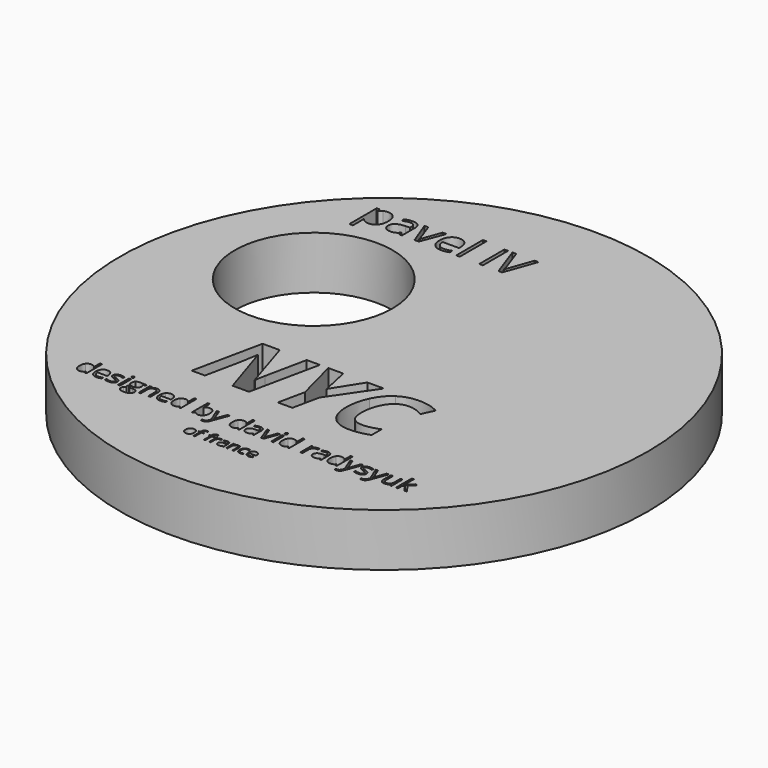
from build123d import *

# Parameters (mm, degrees)
F0_R     = 38.1
F0_W     = 0.3042923246
F0_H     = 2.0080948204
F0_R_2   = 11.3842242746
F0_W_2   = 0.5276449925
F0_H_2   = 4.5401317712
F0_W_3   = 0.5157208118
F0_H_3   = 4.8322741964
F1_DEPTH = 7.62


with BuildPart() as f1:
    # F0 (on Top) → F1 (new body)
    with BuildSketch(Plane.XY):
        Circle(F0_R)
        with BuildLine():
            Line((-23.50456242, -24.6382634649), (-23.5450174689, -24.3691494437))
            Line((-23.5450174689, -24.3691494437), (-23.5614340105, -24.3691494437))
            add(Edge.make_bspline(
                [(-23.5614340105, -24.3691494437), (-23.771917526, -24.6752006835), (-24.1917119468, -24.6752006835)],
                knots=[0, 0, 0, 1, 1, 1], degree=2))
            add(Edge.make_bspline(
                [(-24.1917119468, -24.6752006835), (-24.5857089452, -24.6752006835), (-24.804693884, -24.4057935097)],
                knots=[0, 0, 0, 1, 1, 1], degree=2))
            add(Edge.make_bspline(
                [(-24.804693884, -24.4057935097), (-25.0236788228, -24.136386336), (-25.0236788228, -23.6397859527)],
                knots=[0, 0, 0, 1, 1, 1], degree=2))
            add(Edge.make_bspline(
                [(-25.0236788228, -23.6397859527), (-25.0236788228, -23.1431855694), (-24.8038144264, -22.8682084977)],
                knots=[0, 0, 0, 1, 1, 1], degree=2))
            add(Edge.make_bspline(
                [(-24.8038144264, -22.8682084977), (-24.58395003, -22.5932314259), (-24.1917119468, -22.5932314259)],
                knots=[0, 0, 0, 1, 1, 1], degree=2))
            add(Edge.make_bspline(
                [(-24.1917119468, -22.5932314259), (-23.7830573221, -22.5932314259), (-23.5649518409, -22.8904880898)],
                knots=[0, 0, 0, 1, 1, 1], degree=2))
            Line((-23.5649518409, -22.8904880898), (-23.5409133335, -22.8904880898))
            Line((-23.5409133335, -22.8904880898), (-23.5538120448, -22.7456707407))
            Line((-23.5538120448, -22.7456707407), (-23.5614340105, -22.604371222))
            Line((-23.5614340105, -22.604371222), (-23.5614340105, -21.7870619725))
            Line((-23.5614340105, -21.7870619725), (-23.2571416859, -21.7870619725))
            Line((-23.2571416859, -21.7870619725), (-23.2571416859, -24.6382634649))
            Line((-23.2571416859, -24.6382634649), (-23.50456242, -24.6382634649))
        make_face(mode=Mode.SUBTRACT)
        with BuildLine():
            add(Edge.make_bspline(
                [(-21.4167301119, -24.6447128205), (-21.5603748508, -24.6752006835), (-21.7638227056, -24.6752006835)],
                knots=[0, 0, 0, 1, 1, 1], degree=2))
            add(Edge.make_bspline(
                [(-21.7638227056, -24.6752006835), (-22.2088282439, -24.6752006835), (-22.4665093165, -24.403741442)],
                knots=[0, 0, 0, 1, 1, 1], degree=2))
            add(Edge.make_bspline(
                [(-22.4665093165, -24.403741442), (-22.7241903891, -24.1322822006), (-22.7241903891, -23.6509257488)],
                knots=[0, 0, 0, 1, 1, 1], degree=2))
            add(Edge.make_bspline(
                [(-22.7241903891, -23.6509257488), (-22.7241903891, -23.1648788565), (-22.4849779258, -22.8790551412)],
                knots=[0, 0, 0, 1, 1, 1], degree=2))
            add(Edge.make_bspline(
                [(-22.4849779258, -22.8790551412), (-22.2457654625, -22.5932314259), (-21.8423875833, -22.5932314259)],
                knots=[0, 0, 0, 1, 1, 1], degree=2))
            add(Edge.make_bspline(
                [(-21.8423875833, -22.5932314259), (-21.4653934316, -22.5932314259), (-21.2455290352, -22.8415316176)],
                knots=[0, 0, 0, 1, 1, 1], degree=2))
            add(Edge.make_bspline(
                [(-21.2455290352, -22.8415316176), (-21.0256646388, -23.0898318092), (-21.0256646388, -23.4967275188)],
                knots=[0, 0, 0, 1, 1, 1], degree=2))
            Line((-21.0256646388, -23.4967275188), (-21.0256646388, -23.6890355775))
            Line((-21.0256646388, -23.6890355775), (-22.4087582684, -23.6890355775))
            add(Edge.make_bspline(
                [(-22.4087582684, -23.6890355775), (-22.3993773875, -24.0425775269), (-22.229935226, -24.2257978572)],
                knots=[0, 0, 0, 1, 1, 1], degree=2))
            add(Edge.make_bspline(
                [(-22.229935226, -24.2257978572), (-22.0604930645, -24.4090181876), (-21.7526829096, -24.4090181876)],
                knots=[0, 0, 0, 1, 1, 1], degree=2))
            add(Edge.make_bspline(
                [(-21.7526829096, -24.4090181876), (-21.428456213, -24.4090181876), (-21.1118514822, -24.2735817194)],
                knots=[0, 0, 0, 1, 1, 1], degree=2))
            Line((-21.1118514822, -24.2735817194), (-21.1118514822, -24.5450409608))
            add(Edge.make_bspline(
                [(-21.1118514822, -24.5450409608), (-21.2730853729, -24.6142249575), (-21.4167301119, -24.6447128205)],
                knots=[0, 0, 0, 1, 1, 1], degree=2))
        make_face(mode=Mode.SUBTRACT)
        with BuildLine():
            add(Edge.make_bspline(
                [(-19.3371060746, -23.7588058793), (-19.2116367924, -23.8907245171), (-19.2116367924, -24.0906545416)],
                knots=[0, 0, 0, 1, 1, 1], degree=2))
            add(Edge.make_bspline(
                [(-19.2116367924, -24.0906545416), (-19.2116367924, -24.3709083589), (-19.4203613927, -24.5230545212)],
                knots=[0, 0, 0, 1, 1, 1], degree=2))
            add(Edge.make_bspline(
                [(-19.4203613927, -24.5230545212), (-19.629085993, -24.6752006835), (-20.0066664497, -24.6752006835)],
                knots=[0, 0, 0, 1, 1, 1], degree=2))
            add(Edge.make_bspline(
                [(-20.0066664497, -24.6752006835), (-20.4059401935, -24.6752006835), (-20.6293224203, -24.5485587911)],
                knots=[0, 0, 0, 1, 1, 1], degree=2))
            Line((-20.6293224203, -24.5485587911), (-20.6293224203, -24.2665460587))
            add(Edge.make_bspline(
                [(-20.6293224203, -24.2665460587), (-20.4845050712, -24.3398341908), (-20.3188738926, -24.3817550024)],
                knots=[0, 0, 0, 1, 1, 1], degree=2))
            add(Edge.make_bspline(
                [(-20.3188738926, -24.3817550024), (-20.153242714, -24.423675814), (-19.999044484, -24.423675814)],
                knots=[0, 0, 0, 1, 1, 1], degree=2))
            add(Edge.make_bspline(
                [(-19.999044484, -24.423675814), (-19.7610046308, -24.423675814), (-19.6328969758, -24.3477493091)],
                knots=[0, 0, 0, 1, 1, 1], degree=2))
            add(Edge.make_bspline(
                [(-19.6328969758, -24.3477493091), (-19.5047893209, -24.2718228042), (-19.5047893209, -24.115865659)],
                knots=[0, 0, 0, 1, 1, 1], degree=2))
            add(Edge.make_bspline(
                [(-19.5047893209, -24.115865659), (-19.5047893209, -23.9986046476), (-19.6062200957, -23.9153493295)],
                knots=[0, 0, 0, 1, 1, 1], degree=2))
            add(Edge.make_bspline(
                [(-19.6062200957, -23.9153493295), (-19.7076508706, -23.8320940114), (-20.0031486194, -23.7183508304)],
                knots=[0, 0, 0, 1, 1, 1], degree=2))
            add(Edge.make_bspline(
                [(-20.0031486194, -23.7183508304), (-20.2834024366, -23.6139885302), (-20.4015429056, -23.5360099576)],
                knots=[0, 0, 0, 1, 1, 1], degree=2))
            add(Edge.make_bspline(
                [(-20.4015429056, -23.5360099576), (-20.5196833746, -23.458031385), (-20.5774344227, -23.3592389829)],
                knots=[0, 0, 0, 1, 1, 1], degree=2))
            add(Edge.make_bspline(
                [(-20.5774344227, -23.3592389829), (-20.6351854708, -23.2604465808), (-20.6351854708, -23.1232511975)],
                knots=[0, 0, 0, 1, 1, 1], degree=2))
            add(Edge.make_bspline(
                [(-20.6351854708, -23.1232511975), (-20.6351854708, -22.8775893786), (-20.4352554464, -22.7354104022)],
                knots=[0, 0, 0, 1, 1, 1], degree=2))
            add(Edge.make_bspline(
                [(-20.4352554464, -22.7354104022), (-20.2353254219, -22.5932314259), (-19.8876465231, -22.5932314259)],
                knots=[0, 0, 0, 1, 1, 1], degree=2))
            add(Edge.make_bspline(
                [(-19.8876465231, -22.5932314259), (-19.5634198266, -22.5932314259), (-19.2532644514, -22.7251500637)],
                knots=[0, 0, 0, 1, 1, 1], degree=2))
            Line((-19.2532644514, -22.7251500637), (-19.361730887, -22.9725707978))
            add(Edge.make_bspline(
                [(-19.361730887, -22.9725707978), (-19.6636779913, -22.8482741257), (-19.9093398102, -22.8482741257)],
                knots=[0, 0, 0, 1, 1, 1], degree=2))
            add(Edge.make_bspline(
                [(-19.9093398102, -22.8482741257), (-20.1256863763, -22.8482741257), (-20.2356185745, -22.9159923598)],
                knots=[0, 0, 0, 1, 1, 1], degree=2))
            add(Edge.make_bspline(
                [(-20.2356185745, -22.9159923598), (-20.3455507727, -22.9837105939), (-20.3455507727, -23.1027305205)],
                knots=[0, 0, 0, 1, 1, 1], degree=2))
            add(Edge.make_bspline(
                [(-20.3455507727, -23.1027305205), (-20.3455507727, -23.1836406183), (-20.3042162661, -23.2402190564)],
                knots=[0, 0, 0, 1, 1, 1], degree=2))
            add(Edge.make_bspline(
                [(-20.3042162661, -23.2402190564), (-20.2628817596, -23.2967974944), (-20.1714181707, -23.3480991868)],
                knots=[0, 0, 0, 1, 1, 1], degree=2))
            add(Edge.make_bspline(
                [(-20.1714181707, -23.3480991868), (-20.0799545818, -23.3994008793), (-19.8196351365, -23.4967275188)],
                knots=[0, 0, 0, 1, 1, 1], degree=2))
            add(Edge.make_bspline(
                [(-19.8196351365, -23.4967275188), (-19.4625753568, -23.6268872415), (-19.3371060746, -23.7588058793)],
                knots=[0, 0, 0, 1, 1, 1], degree=2))
        make_face(mode=Mode.SUBTRACT)
        with BuildLine():
            Line((-16.8183395495, -22.6301686445), (-16.124154362, -22.6301686445))
            Line((-16.124154362, -22.6301686445), (-16.124154362, -22.8224767032))
            Line((-16.124154362, -22.8224767032), (-16.4958717681, -22.8664495825))
            add(Edge.make_bspline(
                [(-16.4958717681, -22.8664495825), (-16.4448632282, -22.9303568337), (-16.4044081792, -23.0341328288)],
                knots=[0, 0, 0, 1, 1, 1], degree=2))
            add(Edge.make_bspline(
                [(-16.4044081792, -23.0341328288), (-16.3639531303, -23.1379088239), (-16.3639531303, -23.2674822415)],
                knots=[0, 0, 0, 1, 1, 1], degree=2))
            add(Edge.make_bspline(
                [(-16.3639531303, -23.2674822415), (-16.3639531303, -23.5629799903), (-16.5656420699, -23.7388715074)],
                knots=[0, 0, 0, 1, 1, 1], degree=2))
            add(Edge.make_bspline(
                [(-16.5656420699, -23.7388715074), (-16.7673310096, -23.9147630245), (-17.1191140438, -23.9147630245)],
                knots=[0, 0, 0, 1, 1, 1], degree=2))
            add(Edge.make_bspline(
                [(-17.1191140438, -23.9147630245), (-17.2088187175, -23.9147630245), (-17.2873835951, -23.9001053981)],
                knots=[0, 0, 0, 1, 1, 1], degree=2))
            add(Edge.make_bspline(
                [(-17.2873835951, -23.9001053981), (-17.481450569, -24.002708783), (-17.481450569, -24.1580796231)],
                knots=[0, 0, 0, 1, 1, 1], degree=2))
            add(Edge.make_bspline(
                [(-17.481450569, -24.1580796231), (-17.481450569, -24.2407486362), (-17.4137323349, -24.280031075)],
                knots=[0, 0, 0, 1, 1, 1], degree=2))
            add(Edge.make_bspline(
                [(-17.4137323349, -24.280031075), (-17.3460141009, -24.3193135138), (-17.1812623798, -24.3193135138)],
                knots=[0, 0, 0, 1, 1, 1], degree=2))
            Line((-17.1812623798, -24.3193135138), (-16.8259615153, -24.3193135138))
            add(Edge.make_bspline(
                [(-16.8259615153, -24.3193135138), (-16.4993895985, -24.3193135138), (-16.3246706915, -24.4568020497)],
                knots=[0, 0, 0, 1, 1, 1], degree=2))
            add(Edge.make_bspline(
                [(-16.3246706915, -24.4568020497), (-16.1499517845, -24.5942905856), (-16.1499517845, -24.8563689461)],
                knots=[0, 0, 0, 1, 1, 1], degree=2))
            add(Edge.make_bspline(
                [(-16.1499517845, -24.8563689461), (-16.1499517845, -25.1899765235), (-16.4173068905, -25.3649885831)],
                knots=[0, 0, 0, 1, 1, 1], degree=2))
            add(Edge.make_bspline(
                [(-16.4173068905, -25.3649885831), (-16.6846619965, -25.5400006426), (-17.1976789214, -25.5400006426)],
                knots=[0, 0, 0, 1, 1, 1], degree=2))
            add(Edge.make_bspline(
                [(-17.1976789214, -25.5400006426), (-17.5916759198, -25.5400006426), (-17.8050909605, -25.3934243783)],
                knots=[0, 0, 0, 1, 1, 1], degree=2))
            add(Edge.make_bspline(
                [(-17.8050909605, -25.3934243783), (-18.0185060013, -25.2468481141), (-18.0185060013, -24.978906703)],
                knots=[0, 0, 0, 1, 1, 1], degree=2))
            add(Edge.make_bspline(
                [(-18.0185060013, -24.978906703), (-18.0185060013, -24.7959795252), (-17.9012449899, -24.6620088197)],
                knots=[0, 0, 0, 1, 1, 1], degree=2))
            add(Edge.make_bspline(
                [(-17.9012449899, -24.6620088197), (-17.7839839785, -24.5280381141), (-17.5717415478, -24.4805474045)],
                knots=[0, 0, 0, 1, 1, 1], degree=2))
            add(Edge.make_bspline(
                [(-17.5717415478, -24.4805474045), (-17.6485475103, -24.4459554062), (-17.7007286604, -24.372667274)],
                knots=[0, 0, 0, 1, 1, 1], degree=2))
            add(Edge.make_bspline(
                [(-17.7007286604, -24.372667274), (-17.7529098104, -24.2993791419), (-17.7529098104, -24.2020525024)],
                knots=[0, 0, 0, 1, 1, 1], degree=2))
            add(Edge.make_bspline(
                [(-17.7529098104, -24.2020525024), (-17.7529098104, -24.0924134568), (-17.6942793047, -24.0097444437)],
                knots=[0, 0, 0, 1, 1, 1], degree=2))
            add(Edge.make_bspline(
                [(-17.6942793047, -24.0097444437), (-17.635648799, -23.9270754307), (-17.5090069067, -23.8502694682)],
                knots=[0, 0, 0, 1, 1, 1], degree=2))
            add(Edge.make_bspline(
                [(-17.5090069067, -23.8502694682), (-17.6649640519, -23.786362217), (-17.7628769964, -23.6324571395)],
                knots=[0, 0, 0, 1, 1, 1], degree=2))
            add(Edge.make_bspline(
                [(-17.7628769964, -23.6324571395), (-17.8607899409, -23.478552062), (-17.8607899409, -23.2803809528)],
                knots=[0, 0, 0, 1, 1, 1], degree=2))
            add(Edge.make_bspline(
                [(-17.8607899409, -23.2803809528), (-17.8607899409, -22.9508775107), (-17.6629119842, -22.7720544683)],
                knots=[0, 0, 0, 1, 1, 1], degree=2))
            add(Edge.make_bspline(
                [(-17.6629119842, -22.7720544683), (-17.4650340274, -22.5932314259), (-17.1026975022, -22.5932314259)],
                knots=[0, 0, 0, 1, 1, 1], degree=2))
            add(Edge.make_bspline(
                [(-17.1026975022, -22.5932314259), (-16.9449814418, -22.5932314259), (-16.8183395495, -22.6301686445)],
                knots=[0, 0, 0, 1, 1, 1], degree=2))
        make_face(mode=Mode.SUBTRACT)
        with Locations((-18.5646491619, -23.6342160547)):
            Rectangle(F0_W, F0_H, mode=Mode.SUBTRACT)
        with BuildLine():
            add(Edge.make_bspline(
                [(-18.6912910542, -22.2391031715), (-18.7425927467, -22.1886809366), (-18.7425927467, -22.0860775516)],
                knots=[0, 0, 0, 1, 1, 1], degree=2))
            add(Edge.make_bspline(
                [(-18.7425927467, -22.0860775516), (-18.7425927467, -21.9817152514), (-18.6912910542, -21.9330519317)],
                knots=[0, 0, 0, 1, 1, 1], degree=2))
            add(Edge.make_bspline(
                [(-18.6912910542, -21.9330519317), (-18.6399893617, -21.884388612), (-18.5625970942, -21.884388612)],
                knots=[0, 0, 0, 1, 1, 1], degree=2))
            add(Edge.make_bspline(
                [(-18.5625970942, -21.884388612), (-18.4893089621, -21.884388612), (-18.4362483544, -21.9339313893)],
                knots=[0, 0, 0, 1, 1, 1], degree=2))
            add(Edge.make_bspline(
                [(-18.4362483544, -21.9339313893), (-18.3831877468, -21.9834741666), (-18.3831877468, -22.0860775516)],
                knots=[0, 0, 0, 1, 1, 1], degree=2))
            add(Edge.make_bspline(
                [(-18.3831877468, -22.0860775516), (-18.3831877468, -22.1886809366), (-18.4362483544, -22.2391031715)],
                knots=[0, 0, 0, 1, 1, 1], degree=2))
            add(Edge.make_bspline(
                [(-18.4362483544, -22.2391031715), (-18.4893089621, -22.2895254064), (-18.5625970942, -22.2895254064)],
                knots=[0, 0, 0, 1, 1, 1], degree=2))
            add(Edge.make_bspline(
                [(-18.5625970942, -22.2895254064), (-18.6399893617, -22.2895254064), (-18.6912910542, -22.2391031715)],
                knots=[0, 0, 0, 1, 1, 1], degree=2))
        make_face(mode=Mode.SUBTRACT)
        with BuildLine():
            Line((-14.0333905286, -24.6382634649), (-14.3376828532, -24.6382634649))
            Line((-14.3376828532, -24.6382634649), (-14.3376828532, -23.3390114585))
            add(Edge.make_bspline(
                [(-14.3376828532, -23.3390114585), (-14.3376828532, -23.0939359446), (-14.4493739666, -22.9728639503)],
                knots=[0, 0, 0, 1, 1, 1], degree=2))
            add(Edge.make_bspline(
                [(-14.4493739666, -22.9728639503), (-14.5610650799, -22.8517919561), (-14.7996912381, -22.8517919561)],
                knots=[0, 0, 0, 1, 1, 1], degree=2))
            add(Edge.make_bspline(
                [(-14.7996912381, -22.8517919561), (-15.1145370538, -22.8517919561), (-15.261113318, -23.0221135751)],
                knots=[0, 0, 0, 1, 1, 1], degree=2))
            add(Edge.make_bspline(
                [(-15.261113318, -23.0221135751), (-15.4076895823, -23.1924351942), (-15.4076895823, -23.5846732774)],
                knots=[0, 0, 0, 1, 1, 1], degree=2))
            Line((-15.4076895823, -23.5846732774), (-15.4076895823, -24.6382634649))
            Line((-15.4076895823, -24.6382634649), (-15.7119819069, -24.6382634649))
            Line((-15.7119819069, -24.6382634649), (-15.7119819069, -22.6301686445))
            Line((-15.7119819069, -22.6301686445), (-15.4645611728, -22.6301686445))
            Line((-15.4645611728, -22.6301686445), (-15.415311548, -22.9051457163))
            Line((-15.415311548, -22.9051457163), (-15.4006539216, -22.9051457163))
            add(Edge.make_bspline(
                [(-15.4006539216, -22.9051457163), (-15.3068451125, -22.7568105368), (-15.1382824086, -22.6750209814)],
                knots=[0, 0, 0, 1, 1, 1], degree=2))
            add(Edge.make_bspline(
                [(-15.1382824086, -22.6750209814), (-14.9697197047, -22.5932314259), (-14.7627540195, -22.5932314259)],
                knots=[0, 0, 0, 1, 1, 1], degree=2))
            add(Edge.make_bspline(
                [(-14.7627540195, -22.5932314259), (-14.3998311892, -22.5932314259), (-14.2166108589, -22.7682434854)],
                knots=[0, 0, 0, 1, 1, 1], degree=2))
            add(Edge.make_bspline(
                [(-14.2166108589, -22.7682434854), (-14.0333905286, -22.943255545), (-14.0333905286, -23.3284579674)],
                knots=[0, 0, 0, 1, 1, 1], degree=2))
            Line((-14.0333905286, -23.3284579674), (-14.0333905286, -24.6382634649))
        make_face(mode=Mode.SUBTRACT)
        with BuildLine():
            add(Edge.make_bspline(
                [(-12.2134996315, -24.6447128205), (-12.3571443705, -24.6752006835), (-12.5605922253, -24.6752006835)],
                knots=[0, 0, 0, 1, 1, 1], degree=2))
            add(Edge.make_bspline(
                [(-12.5605922253, -24.6752006835), (-13.0055977636, -24.6752006835), (-13.2632788362, -24.403741442)],
                knots=[0, 0, 0, 1, 1, 1], degree=2))
            add(Edge.make_bspline(
                [(-13.2632788362, -24.403741442), (-13.5209599087, -24.1322822006), (-13.5209599087, -23.6509257488)],
                knots=[0, 0, 0, 1, 1, 1], degree=2))
            add(Edge.make_bspline(
                [(-13.5209599087, -23.6509257488), (-13.5209599087, -23.1648788565), (-13.2817474455, -22.8790551412)],
                knots=[0, 0, 0, 1, 1, 1], degree=2))
            add(Edge.make_bspline(
                [(-13.2817474455, -22.8790551412), (-13.0425349822, -22.5932314259), (-12.6391571029, -22.5932314259)],
                knots=[0, 0, 0, 1, 1, 1], degree=2))
            add(Edge.make_bspline(
                [(-12.6391571029, -22.5932314259), (-12.2621629513, -22.5932314259), (-12.0422985549, -22.8415316176)],
                knots=[0, 0, 0, 1, 1, 1], degree=2))
            add(Edge.make_bspline(
                [(-12.0422985549, -22.8415316176), (-11.8224341585, -23.0898318092), (-11.8224341585, -23.4967275188)],
                knots=[0, 0, 0, 1, 1, 1], degree=2))
            Line((-11.8224341585, -23.4967275188), (-11.8224341585, -23.6890355775))
            Line((-11.8224341585, -23.6890355775), (-13.205527788, -23.6890355775))
            add(Edge.make_bspline(
                [(-13.205527788, -23.6890355775), (-13.1961469071, -24.0425775269), (-13.0267047456, -24.2257978572)],
                knots=[0, 0, 0, 1, 1, 1], degree=2))
            add(Edge.make_bspline(
                [(-13.0267047456, -24.2257978572), (-12.8572625842, -24.4090181876), (-12.5494524292, -24.4090181876)],
                knots=[0, 0, 0, 1, 1, 1], degree=2))
            add(Edge.make_bspline(
                [(-12.5494524292, -24.4090181876), (-12.2252257327, -24.4090181876), (-11.9086210019, -24.2735817194)],
                knots=[0, 0, 0, 1, 1, 1], degree=2))
            Line((-11.9086210019, -24.2735817194), (-11.9086210019, -24.5450409608))
            add(Edge.make_bspline(
                [(-11.9086210019, -24.5450409608), (-12.0698548926, -24.6142249575), (-12.2134996315, -24.6447128205)],
                knots=[0, 0, 0, 1, 1, 1], degree=2))
        make_face(mode=Mode.SUBTRACT)
        with BuildLine():
            Line((-9.8964220461, -24.6382634649), (-9.936877095, -24.3691494437))
            Line((-9.936877095, -24.3691494437), (-9.9532936366, -24.3691494437))
            add(Edge.make_bspline(
                [(-9.9532936366, -24.3691494437), (-10.1637771521, -24.6752006835), (-10.583571573, -24.6752006835)],
                knots=[0, 0, 0, 1, 1, 1], degree=2))
            add(Edge.make_bspline(
                [(-10.583571573, -24.6752006835), (-10.9775685713, -24.6752006835), (-11.1965535101, -24.4057935097)],
                knots=[0, 0, 0, 1, 1, 1], degree=2))
            add(Edge.make_bspline(
                [(-11.1965535101, -24.4057935097), (-11.4155384489, -24.136386336), (-11.4155384489, -23.6397859527)],
                knots=[0, 0, 0, 1, 1, 1], degree=2))
            add(Edge.make_bspline(
                [(-11.4155384489, -23.6397859527), (-11.4155384489, -23.1431855694), (-11.1956740525, -22.8682084977)],
                knots=[0, 0, 0, 1, 1, 1], degree=2))
            add(Edge.make_bspline(
                [(-11.1956740525, -22.8682084977), (-10.9758096561, -22.5932314259), (-10.583571573, -22.5932314259)],
                knots=[0, 0, 0, 1, 1, 1], degree=2))
            add(Edge.make_bspline(
                [(-10.583571573, -22.5932314259), (-10.1749169482, -22.5932314259), (-9.956811467, -22.8904880898)],
                knots=[0, 0, 0, 1, 1, 1], degree=2))
            Line((-9.956811467, -22.8904880898), (-9.9327729596, -22.8904880898))
            Line((-9.9327729596, -22.8904880898), (-9.9456716709, -22.7456707407))
            Line((-9.9456716709, -22.7456707407), (-9.9532936366, -22.604371222))
            Line((-9.9532936366, -22.604371222), (-9.9532936366, -21.7870619725))
            Line((-9.9532936366, -21.7870619725), (-9.649001312, -21.7870619725))
            Line((-9.649001312, -21.7870619725), (-9.649001312, -24.6382634649))
            Line((-9.649001312, -24.6382634649), (-9.8964220461, -24.6382634649))
        make_face(mode=Mode.SUBTRACT)
        with BuildLine():
            add(Edge.make_bspline(
                [(-4.8760077284, -27.8593197968), (-4.70989281, -28.0470080813), (-4.70989281, -28.3666861416)],
                knots=[0, 0, 0, 1, 1, 1], degree=2))
            add(Edge.make_bspline(
                [(-4.70989281, -28.3666861416), (-4.70989281, -28.6953857914), (-4.8752232424, -28.8799361318)],
                knots=[0, 0, 0, 1, 1, 1], degree=2))
            add(Edge.make_bspline(
                [(-4.8752232424, -28.8799361318), (-5.0405536748, -29.0644864722), (-5.3323824809, -29.0644864722)],
                knots=[0, 0, 0, 1, 1, 1], degree=2))
            add(Edge.make_bspline(
                [(-5.3323824809, -29.0644864722), (-5.5128142695, -29.0644864722), (-5.6524527842, -28.9797619801)],
                knots=[0, 0, 0, 1, 1, 1], degree=2))
            add(Edge.make_bspline(
                [(-5.6524527842, -28.9797619801), (-5.7920912989, -28.895037488), (-5.8681864446, -28.7369635514)],
                knots=[0, 0, 0, 1, 1, 1], degree=2))
            add(Edge.make_bspline(
                [(-5.8681864446, -28.7369635514), (-5.9442815903, -28.5788896148), (-5.9442815903, -28.3666861416)],
                knots=[0, 0, 0, 1, 1, 1], degree=2))
            add(Edge.make_bspline(
                [(-5.9442815903, -28.3666861416), (-5.9442815903, -28.0383787349), (-5.7799317654, -27.8550051236)],
                knots=[0, 0, 0, 1, 1, 1], degree=2))
            add(Edge.make_bspline(
                [(-5.7799317654, -27.8550051236), (-5.6155819405, -27.6716315123), (-5.3237531344, -27.6716315123)],
                knots=[0, 0, 0, 1, 1, 1], degree=2))
            add(Edge.make_bspline(
                [(-5.3237531344, -27.6716315123), (-5.0421226469, -27.6716315123), (-4.8760077284, -27.8593197968)],
                knots=[0, 0, 0, 1, 1, 1], degree=2))
        make_face(mode=Mode.SUBTRACT)
        with BuildLine():
            Line((-5.2382283679, -24.6494032609), (-6.0485019568, -22.6301686445))
            Line((-6.0485019568, -22.6301686445), (-5.72193004, -22.6301686445))
            Line((-5.72193004, -22.6301686445), (-5.2822012472, -23.7752224209))
            add(Edge.make_bspline(
                [(-5.2822012472, -23.7752224209), (-5.1379702032, -24.1674605041), (-5.1027918998, -24.341593106)],
                knots=[0, 0, 0, 1, 1, 1], degree=2))
            Line((-5.1027918998, -24.341593106), (-5.0881342733, -24.341593106))
            add(Edge.make_bspline(
                [(-5.0881342733, -24.341593106), (-5.0646820711, -24.2477842969), (-4.9884624136, -24.0214705449)],
                knots=[0, 0, 0, 1, 1, 1], degree=2))
            add(Edge.make_bspline(
                [(-4.9884624136, -24.0214705449), (-4.9122427562, -23.7951567928), (-4.4906894202, -22.6301686445)],
                knots=[0, 0, 0, 1, 1, 1], degree=2))
            Line((-4.4906894202, -22.6301686445), (-4.1647038085, -22.6301686445))
            Line((-4.1647038085, -22.6301686445), (-5.0277448525, -24.916758367))
            add(Edge.make_bspline(
                [(-5.0277448525, -24.916758367), (-5.15614566, -25.2556426899), (-5.3273467366, -25.3978216663)],
                knots=[0, 0, 0, 1, 1, 1], degree=2))
            add(Edge.make_bspline(
                [(-5.3273467366, -25.3978216663), (-5.4985478133, -25.5400006426), (-5.7477274625, -25.5400006426)],
                knots=[0, 0, 0, 1, 1, 1], degree=2))
            add(Edge.make_bspline(
                [(-5.7477274625, -25.5400006426), (-5.8872680661, -25.5400006426), (-6.0227045343, -25.5083401695)],
                knots=[0, 0, 0, 1, 1, 1], degree=2))
            Line((-6.0227045343, -25.5083401695), (-6.0227045343, -25.2650235708))
            add(Edge.make_bspline(
                [(-6.0227045343, -25.2650235708), (-5.9218600644, -25.2867168579), (-5.7975633924, -25.2867168579)],
                knots=[0, 0, 0, 1, 1, 1], degree=2))
            add(Edge.make_bspline(
                [(-5.7975633924, -25.2867168579), (-5.4838901868, -25.2867168579), (-5.3502126338, -24.9349338237)],
                knots=[0, 0, 0, 1, 1, 1], degree=2))
            Line((-5.3502126338, -24.9349338237), (-5.2382283679, -24.6494032609))
        make_face(mode=Mode.SUBTRACT)
        with BuildLine():
            Line((-3.7473284417, -27.6963428224), (-3.7473284417, -27.854416759))
            Line((-3.7473284417, -27.854416759), (-4.0893643541, -27.854416759))
            Line((-4.0893643541, -27.854416759), (-4.0893643541, -29.039775162))
            Line((-4.0893643541, -29.039775162), (-4.2929384809, -29.039775162))
            Line((-4.2929384809, -29.039775162), (-4.2929384809, -27.854416759))
            Line((-4.2929384809, -27.854416759), (-4.5329912085, -27.854416759))
            Line((-4.5329912085, -27.854416759), (-4.5329912085, -27.7626318926))
            Line((-4.5329912085, -27.7626318926), (-4.2929384809, -27.6888902051))
            Line((-4.2929384809, -27.6888902051), (-4.2929384809, -27.6143640315))
            add(Edge.make_bspline(
                [(-4.2929384809, -27.6143640315), (-4.2929384809, -27.1189610987), (-3.8602944311, -27.1189610987)],
                knots=[0, 0, 0, 1, 1, 1], degree=2))
            add(Edge.make_bspline(
                [(-3.8602944311, -27.1189610987), (-3.75360433, -27.1189610987), (-3.6100433851, -27.1617155878)],
                knots=[0, 0, 0, 1, 1, 1], degree=2))
            Line((-3.6100433851, -27.1617155878), (-3.6629961927, -27.3248886836))
            add(Edge.make_bspline(
                [(-3.6629961927, -27.3248886836), (-3.7806690983, -27.2868411108), (-3.8638246183, -27.2868411108)],
                knots=[0, 0, 0, 1, 1, 1], degree=2))
            add(Edge.make_bspline(
                [(-3.8638246183, -27.2868411108), (-3.9791440659, -27.2868411108), (-4.03425421, -27.363524621)],
                knots=[0, 0, 0, 1, 1, 1], degree=2))
            add(Edge.make_bspline(
                [(-4.03425421, -27.363524621), (-4.0893643541, -27.4402081311), (-4.0893643541, -27.6092648723)],
                knots=[0, 0, 0, 1, 1, 1], degree=2))
            Line((-4.0893643541, -27.6092648723), (-4.0893643541, -27.6963428224))
            Line((-4.0893643541, -27.6963428224), (-3.7473284417, -27.6963428224))
        make_face(mode=Mode.SUBTRACT)
        with BuildLine():
            Line((-2.2442531935, -27.6963428224), (-2.2442531935, -27.854416759))
            Line((-2.2442531935, -27.854416759), (-2.5862891059, -27.854416759))
            Line((-2.5862891059, -27.854416759), (-2.5862891059, -29.039775162))
            Line((-2.5862891059, -29.039775162), (-2.7898632327, -29.039775162))
            Line((-2.7898632327, -29.039775162), (-2.7898632327, -27.854416759))
            Line((-2.7898632327, -27.854416759), (-3.0299159603, -27.854416759))
            Line((-3.0299159603, -27.854416759), (-3.0299159603, -27.7626318926))
            Line((-3.0299159603, -27.7626318926), (-2.7898632327, -27.6888902051))
            Line((-2.7898632327, -27.6888902051), (-2.7898632327, -27.6143640315))
            add(Edge.make_bspline(
                [(-2.7898632327, -27.6143640315), (-2.7898632327, -27.1189610987), (-2.3572191829, -27.1189610987)],
                knots=[0, 0, 0, 1, 1, 1], degree=2))
            add(Edge.make_bspline(
                [(-2.3572191829, -27.1189610987), (-2.2505290818, -27.1189610987), (-2.1069681369, -27.1617155878)],
                knots=[0, 0, 0, 1, 1, 1], degree=2))
            Line((-2.1069681369, -27.1617155878), (-2.1599209445, -27.3248886836))
            add(Edge.make_bspline(
                [(-2.1599209445, -27.3248886836), (-2.2775938501, -27.2868411108), (-2.3607493701, -27.2868411108)],
                knots=[0, 0, 0, 1, 1, 1], degree=2))
            add(Edge.make_bspline(
                [(-2.3607493701, -27.2868411108), (-2.4760688176, -27.2868411108), (-2.5311789618, -27.363524621)],
                knots=[0, 0, 0, 1, 1, 1], degree=2))
            add(Edge.make_bspline(
                [(-2.5311789618, -27.363524621), (-2.5862891059, -27.4402081311), (-2.5862891059, -27.6092648723)],
                knots=[0, 0, 0, 1, 1, 1], degree=2))
            Line((-2.5862891059, -27.6092648723), (-2.5862891059, -27.6963428224))
            Line((-2.5862891059, -27.6963428224), (-2.2442531935, -27.6963428224))
        make_face(mode=Mode.SUBTRACT)
        with BuildLine():
            add(Edge.make_bspline(
                [(-1.6178410924, -27.7428236202), (-1.5123277204, -27.6716315123), (-1.3860254683, -27.6716315123)],
                knots=[0, 0, 0, 1, 1, 1], degree=2))
            add(Edge.make_bspline(
                [(-1.3860254683, -27.6716315123), (-1.29659406, -27.6716315123), (-1.2255980736, -27.686536747)],
                knots=[0, 0, 0, 1, 1, 1], degree=2))
            Line((-1.2255980736, -27.686536747), (-1.2538395709, -27.875205639))
            add(Edge.make_bspline(
                [(-1.2538395709, -27.875205639), (-1.3369950909, -27.8567702172), (-1.400930703, -27.8567702172)],
                knots=[0, 0, 0, 1, 1, 1], degree=2))
            add(Edge.make_bspline(
                [(-1.400930703, -27.8567702172), (-1.5641037988, -27.8567702172), (-1.6798154894, -27.989152236)],
                knots=[0, 0, 0, 1, 1, 1], degree=2))
            add(Edge.make_bspline(
                [(-1.6798154894, -27.989152236), (-1.79552718, -28.1215342549), (-1.79552718, -28.3188324933)],
                knots=[0, 0, 0, 1, 1, 1], degree=2))
            Line((-1.79552718, -28.3188324933), (-1.79552718, -29.039775162))
            Line((-1.79552718, -29.039775162), (-1.9991013067, -29.039775162))
            Line((-1.9991013067, -29.039775162), (-1.9991013067, -27.6963428224))
            Line((-1.9991013067, -27.6963428224), (-1.8312212947, -27.6963428224))
            Line((-1.8312212947, -27.6963428224), (-1.8076867135, -27.9450248964))
            Line((-1.8076867135, -27.9450248964), (-1.7978806381, -27.9450248964))
            add(Edge.make_bspline(
                [(-1.7978806381, -27.9450248964), (-1.7233544645, -27.8140157281), (-1.6178410924, -27.7428236202)],
                knots=[0, 0, 0, 1, 1, 1], degree=2))
        make_face(mode=Mode.SUBTRACT)
        with BuildLine():
            Line((0.0029070614, -29.039775162), (-0.1481065008, -29.039775162))
            Line((-0.1481065008, -29.039775162), (-0.1885075318, -28.8483605688))
            Line((-0.1885075318, -28.8483605688), (-0.1983136072, -28.8483605688))
            add(Edge.make_bspline(
                [(-0.1983136072, -28.8483605688), (-0.2987278201, -28.9746628209), (-0.3985536683, -29.0195746465)],
                knots=[0, 0, 0, 1, 1, 1], degree=2))
            add(Edge.make_bspline(
                [(-0.3985536683, -29.0195746465), (-0.4983795166, -29.0644864722), (-0.6482163498, -29.0644864722)],
                knots=[0, 0, 0, 1, 1, 1], degree=2))
            add(Edge.make_bspline(
                [(-0.6482163498, -29.0644864722), (-0.8478680464, -29.0644864722), (-0.9612262789, -28.9613265582)],
                knots=[0, 0, 0, 1, 1, 1], degree=2))
            add(Edge.make_bspline(
                [(-0.9612262789, -28.9613265582), (-1.0745845113, -28.8581666443), (-1.0745845113, -28.6683210231)],
                knots=[0, 0, 0, 1, 1, 1], degree=2))
            add(Edge.make_bspline(
                [(-1.0745845113, -28.6683210231), (-1.0745845113, -28.2615650126), (-0.4238533431, -28.2419528617)],
                knots=[0, 0, 0, 1, 1, 1], degree=2))
            Line((-0.4238533431, -28.2419528617), (-0.1959601491, -28.2345002443))
            Line((-0.1959601491, -28.2345002443), (-0.1959601491, -28.1509524813))
            add(Edge.make_bspline(
                [(-0.1959601491, -28.1509524813), (-0.1959601491, -27.9928785447), (-0.2638181914, -27.9175678851)],
                knots=[0, 0, 0, 1, 1, 1], degree=2))
            add(Edge.make_bspline(
                [(-0.2638181914, -27.9175678851), (-0.3316762336, -27.8422572255), (-0.4815130668, -27.8422572255)],
                knots=[0, 0, 0, 1, 1, 1], degree=2))
            add(Edge.make_bspline(
                [(-0.4815130668, -27.8422572255), (-0.6493930789, -27.8422572255), (-0.8612043091, -27.9450248964)],
                knots=[0, 0, 0, 1, 1, 1], degree=2))
            Line((-0.8612043091, -27.9450248964), (-0.9239631921, -27.7893044179))
            add(Edge.make_bspline(
                [(-0.9239631921, -27.7893044179), (-0.8247257083, -27.7355671243), (-0.7064644381, -27.7049721689)],
                knots=[0, 0, 0, 1, 1, 1], degree=2))
            add(Edge.make_bspline(
                [(-0.7064644381, -27.7049721689), (-0.588203168, -27.6743772134), (-0.4689612902, -27.6743772134)],
                knots=[0, 0, 0, 1, 1, 1], degree=2))
            add(Edge.make_bspline(
                [(-0.4689612902, -27.6743772134), (-0.2289085627, -27.6743772134), (-0.1130007506, -27.780871193)],
                knots=[0, 0, 0, 1, 1, 1], degree=2))
            add(Edge.make_bspline(
                [(-0.1130007506, -27.780871193), (0.0029070614, -27.8873651726), (0.0029070614, -28.1227109839)],
                knots=[0, 0, 0, 1, 1, 1], degree=2))
            Line((0.0029070614, -28.1227109839), (0.0029070614, -29.039775162))
        make_face(mode=Mode.SUBTRACT)
        with BuildLine():
            add(Edge.make_bspline(
                [(-7.7247481148, -22.8975237505), (-7.5125056842, -22.5973355613), (-7.0944701785, -22.5973355613)],
                knots=[0, 0, 0, 1, 1, 1], degree=2))
            add(Edge.make_bspline(
                [(-7.0944701785, -22.5973355613), (-6.698714265, -22.5973355613), (-6.4797293262, -22.8676221926)],
                knots=[0, 0, 0, 1, 1, 1], degree=2))
            add(Edge.make_bspline(
                [(-6.4797293262, -22.8676221926), (-6.2607443874, -23.1379088239), (-6.2607443874, -23.632163987)],
                knots=[0, 0, 0, 1, 1, 1], degree=2))
            add(Edge.make_bspline(
                [(-6.2607443874, -23.632163987), (-6.2607443874, -24.1270054551), (-6.4814882414, -24.4011030693)],
                knots=[0, 0, 0, 1, 1, 1], degree=2))
            add(Edge.make_bspline(
                [(-6.4814882414, -24.4011030693), (-6.7022320954, -24.6752006835), (-7.0944701785, -24.6752006835)],
                knots=[0, 0, 0, 1, 1, 1], degree=2))
            add(Edge.make_bspline(
                [(-7.0944701785, -24.6752006835), (-7.2908823726, -24.6752006835), (-7.4529957209, -24.6027920089)],
                knots=[0, 0, 0, 1, 1, 1], degree=2))
            add(Edge.make_bspline(
                [(-7.4529957209, -24.6027920089), (-7.6151090692, -24.5303833344), (-7.7247481148, -24.3797029347)],
                knots=[0, 0, 0, 1, 1, 1], degree=2))
            Line((-7.7247481148, -24.3797029347), (-7.747027707, -24.3797029347))
            Line((-7.747027707, -24.3797029347), (-7.8109349582, -24.6382634649))
            Line((-7.8109349582, -24.6382634649), (-8.0290404394, -24.6382634649))
            Line((-8.0290404394, -24.6382634649), (-8.0290404394, -21.7870619725))
            Line((-8.0290404394, -21.7870619725), (-7.7247481148, -21.7870619725))
            Line((-7.7247481148, -21.7870619725), (-7.7247481148, -22.4800745499))
            add(Edge.make_bspline(
                [(-7.7247481148, -22.4800745499), (-7.7247481148, -22.7128376575), (-7.7394057413, -22.8975237505)],
                knots=[0, 0, 0, 1, 1, 1], degree=2))
            Line((-7.7394057413, -22.8975237505), (-7.7247481148, -22.8975237505))
        make_face(mode=Mode.SUBTRACT)
        with BuildLine():
            Line((-1.45656075, -24.6382634649), (-1.497015799, -24.3691494437))
            Line((-1.497015799, -24.3691494437), (-1.5134323406, -24.3691494437))
            add(Edge.make_bspline(
                [(-1.5134323406, -24.3691494437), (-1.723915856, -24.6752006835), (-2.1437102769, -24.6752006835)],
                knots=[0, 0, 0, 1, 1, 1], degree=2))
            add(Edge.make_bspline(
                [(-2.1437102769, -24.6752006835), (-2.5377072752, -24.6752006835), (-2.756692214, -24.4057935097)],
                knots=[0, 0, 0, 1, 1, 1], degree=2))
            add(Edge.make_bspline(
                [(-2.756692214, -24.4057935097), (-2.9756771528, -24.136386336), (-2.9756771528, -23.6397859527)],
                knots=[0, 0, 0, 1, 1, 1], degree=2))
            add(Edge.make_bspline(
                [(-2.9756771528, -23.6397859527), (-2.9756771528, -23.1431855694), (-2.7558127564, -22.8682084977)],
                knots=[0, 0, 0, 1, 1, 1], degree=2))
            add(Edge.make_bspline(
                [(-2.7558127564, -22.8682084977), (-2.53594836, -22.5932314259), (-2.1437102769, -22.5932314259)],
                knots=[0, 0, 0, 1, 1, 1], degree=2))
            add(Edge.make_bspline(
                [(-2.1437102769, -22.5932314259), (-1.7350556521, -22.5932314259), (-1.5169501709, -22.8904880898)],
                knots=[0, 0, 0, 1, 1, 1], degree=2))
            Line((-1.5169501709, -22.8904880898), (-1.4929116636, -22.8904880898))
            Line((-1.4929116636, -22.8904880898), (-1.5058103748, -22.7456707407))
            Line((-1.5058103748, -22.7456707407), (-1.5134323406, -22.604371222))
            Line((-1.5134323406, -22.604371222), (-1.5134323406, -21.7870619725))
            Line((-1.5134323406, -21.7870619725), (-1.209140016, -21.7870619725))
            Line((-1.209140016, -21.7870619725), (-1.209140016, -24.6382634649))
            Line((-1.209140016, -24.6382634649), (-1.45656075, -24.6382634649))
        make_face(mode=Mode.SUBTRACT)
        with BuildLine():
            Line((-3.9886239994, -6.5999108824), (-6.12824639, -16.7199261025))
            Line((-6.12824639, -16.7199261025), (-8.4960065717, -16.7199261025))
            Line((-8.4960065717, -16.7199261025), (-10.9590087439, -9.0651279846))
            Line((-10.9590087439, -9.0651279846), (-11.0010924141, -9.0651279846))
            Line((-11.0010924141, -9.0651279846), (-11.0298865042, -9.2866209857))
            add(Edge.make_bspline(
                [(-11.0298865042, -9.2866209857), (-11.2513795053, -10.7816987431), (-11.4861620865, -11.9578265789)],
                knots=[0, 0, 0, 1, 1, 1], degree=2))
            Line((-11.4861620865, -11.9578265789), (-12.4895253815, -16.7199261025))
            Line((-12.4895253815, -16.7199261025), (-14.3921502609, -16.7199261025))
            Line((-14.3921502609, -16.7199261025), (-12.2547428003, -6.5999108824))
            Line((-12.2547428003, -6.5999108824), (-9.7828809081, -6.5999108824))
            Line((-9.7828809081, -6.5999108824), (-7.4306252364, -14.0553652993))
            Line((-7.4306252364, -14.0553652993), (-7.4018311463, -14.0553652993))
            add(Edge.make_bspline(
                [(-7.4018311463, -14.0553652993), (-7.3198787359, -13.5282119567), (-7.1327171499, -12.5525352868)],
                knots=[0, 0, 0, 1, 1, 1], degree=2))
            add(Edge.make_bspline(
                [(-7.1327171499, -12.5525352868), (-6.945555564, -11.576858617), (-5.8868190188, -6.5999108824)],
                knots=[0, 0, 0, 1, 1, 1], degree=2))
            Line((-5.8868190188, -6.5999108824), (-3.9886239994, -6.5999108824))
        make_face(mode=Mode.SUBTRACT)
        with BuildLine():
            Line((1.5448143685, -29.039775162), (1.3412402417, -29.039775162))
            Line((1.3412402417, -29.039775162), (1.3412402417, -28.1705646322))
            add(Edge.make_bspline(
                [(1.3412402417, -28.1705646322), (1.3412402417, -28.0066070504), (1.2665179466, -27.925608867)],
                knots=[0, 0, 0, 1, 1, 1], degree=2))
            add(Edge.make_bspline(
                [(1.2665179466, -27.925608867), (1.1917956516, -27.8446106836), (1.0321527429, -27.8446106836)],
                knots=[0, 0, 0, 1, 1, 1], degree=2))
            add(Edge.make_bspline(
                [(1.0321527429, -27.8446106836), (0.8215182418, -27.8446106836), (0.7234574871, -27.9585572805)],
                knots=[0, 0, 0, 1, 1, 1], degree=2))
            add(Edge.make_bspline(
                [(0.7234574871, -27.9585572805), (0.6253967323, -28.0725038775), (0.6253967323, -28.3349144571)],
                knots=[0, 0, 0, 1, 1, 1], degree=2))
            Line((0.6253967323, -28.3349144571), (0.6253967323, -29.039775162))
            Line((0.6253967323, -29.039775162), (0.4218226056, -29.039775162))
            Line((0.4218226056, -29.039775162), (0.4218226056, -27.6963428224))
            Line((0.4218226056, -27.6963428224), (0.5873491595, -27.6963428224))
            Line((0.5873491595, -27.6963428224), (0.6202975731, -27.8803047983))
            Line((0.6202975731, -27.8803047983), (0.6301036486, -27.8803047983))
            add(Edge.make_bspline(
                [(0.6301036486, -27.8803047983), (0.6928625316, -27.7810673145), (0.8056323995, -27.7263494134)],
                knots=[0, 0, 0, 1, 1, 1], degree=2))
            add(Edge.make_bspline(
                [(0.8056323995, -27.7263494134), (0.9184022674, -27.6716315123), (1.0568640531, -27.6716315123)],
                knots=[0, 0, 0, 1, 1, 1], degree=2))
            add(Edge.make_bspline(
                [(1.0568640531, -27.6716315123), (1.2996624817, -27.6716315123), (1.4222384251, -27.7887160534)],
                knots=[0, 0, 0, 1, 1, 1], degree=2))
            add(Edge.make_bspline(
                [(1.4222384251, -27.7887160534), (1.5448143685, -27.9058005945), (1.5448143685, -28.1635042579)],
                knots=[0, 0, 0, 1, 1, 1], degree=2))
            Line((1.5448143685, -28.1635042579), (1.5448143685, -29.039775162))
        make_face(mode=Mode.SUBTRACT)
        with BuildLine():
            add(Edge.make_bspline(
                [(2.8388240877, -28.9942749718), (2.7042847322, -29.0644864722), (2.4995338764, -29.0644864722)],
                knots=[0, 0, 0, 1, 1, 1], degree=2))
            add(Edge.make_bspline(
                [(2.4995338764, -29.0644864722), (2.2077050704, -29.0644864722), (2.0476699187, -28.8848391695)],
                knots=[0, 0, 0, 1, 1, 1], degree=2))
            add(Edge.make_bspline(
                [(2.0476699187, -28.8848391695), (1.887634767, -28.7051918669), (1.887634767, -28.3764922171)],
                knots=[0, 0, 0, 1, 1, 1], degree=2))
            add(Edge.make_bspline(
                [(1.887634767, -28.3764922171), (1.887634767, -28.0395554639), (2.0502194983, -27.8555934881)],
                knots=[0, 0, 0, 1, 1, 1], degree=2))
            add(Edge.make_bspline(
                [(2.0502194983, -27.8555934881), (2.2128042296, -27.6716315123), (2.512870139, -27.6716315123)],
                knots=[0, 0, 0, 1, 1, 1], degree=2))
            add(Edge.make_bspline(
                [(2.512870139, -27.6716315123), (2.6097541647, -27.6716315123), (2.7066381903, -27.6926165138)],
                knots=[0, 0, 0, 1, 1, 1], degree=2))
            add(Edge.make_bspline(
                [(2.7066381903, -27.6926165138), (2.803522216, -27.7136015153), (2.8584362386, -27.7418430126)],
                knots=[0, 0, 0, 1, 1, 1], degree=2))
            Line((2.8584362386, -27.7418430126), (2.7960695986, -27.9144299409))
            add(Edge.make_bspline(
                [(2.7960695986, -27.9144299409), (2.7286037994, -27.8873651726), (2.6489784666, -27.8697142368)],
                knots=[0, 0, 0, 1, 1, 1], degree=2))
            add(Edge.make_bspline(
                [(2.6489784666, -27.8697142368), (2.5693531337, -27.8520633009), (2.5081632228, -27.8520633009)],
                knots=[0, 0, 0, 1, 1, 1], degree=2))
            add(Edge.make_bspline(
                [(2.5081632228, -27.8520633009), (2.0986615111, -27.8520633009), (2.0986615111, -28.374138759)],
                knots=[0, 0, 0, 1, 1, 1], degree=2))
            add(Edge.make_bspline(
                [(2.0986615111, -28.374138759), (2.0986615111, -28.6216441039), (2.1984873594, -28.7540261228)],
                knots=[0, 0, 0, 1, 1, 1], degree=2))
            add(Edge.make_bspline(
                [(2.1984873594, -28.7540261228), (2.2983132077, -28.8864081416), (2.4944347171, -28.8864081416)],
                knots=[0, 0, 0, 1, 1, 1], degree=2))
            add(Edge.make_bspline(
                [(2.4944347171, -28.8864081416), (2.6623147292, -28.8864081416), (2.8388240877, -28.8142354261)],
                knots=[0, 0, 0, 1, 1, 1], degree=2))
            Line((2.8388240877, -28.8142354261), (2.8388240877, -28.9942749718))
        make_face(mode=Mode.SUBTRACT)
        with BuildLine():
            add(Edge.make_bspline(
                [(3.9575011774, -29.0440898352), (3.8614016378, -29.0644864722), (3.7252933103, -29.0644864722)],
                knots=[0, 0, 0, 1, 1, 1], degree=2))
            add(Edge.make_bspline(
                [(3.7252933103, -29.0644864722), (3.427580859, -29.0644864722), (3.2551900522, -28.8828779544)],
                knots=[0, 0, 0, 1, 1, 1], degree=2))
            add(Edge.make_bspline(
                [(3.2551900522, -28.8828779544), (3.0827992454, -28.7012694367), (3.0827992454, -28.3792379183)],
                knots=[0, 0, 0, 1, 1, 1], degree=2))
            add(Edge.make_bspline(
                [(3.0827992454, -28.3792379183), (3.0827992454, -28.0540684556), (3.2428343971, -27.8628499839)],
                knots=[0, 0, 0, 1, 1, 1], degree=2))
            add(Edge.make_bspline(
                [(3.2428343971, -27.8628499839), (3.4028695488, -27.6716315123), (3.6727327457, -27.6716315123)],
                knots=[0, 0, 0, 1, 1, 1], degree=2))
            add(Edge.make_bspline(
                [(3.6727327457, -27.6716315123), (3.9249450068, -27.6716315123), (4.0720361389, -27.8377464307)],
                knots=[0, 0, 0, 1, 1, 1], degree=2))
            add(Edge.make_bspline(
                [(4.0720361389, -27.8377464307), (4.219127271, -28.0038613492), (4.219127271, -28.2760780043)],
                knots=[0, 0, 0, 1, 1, 1], degree=2))
            Line((4.219127271, -28.2760780043), (4.219127271, -28.4047337145))
            Line((4.219127271, -28.4047337145), (3.2938259895, -28.4047337145))
            add(Edge.make_bspline(
                [(3.2938259895, -28.4047337145), (3.3001018778, -28.6412562548), (3.4134601103, -28.7638321982)],
                knots=[0, 0, 0, 1, 1, 1], degree=2))
            add(Edge.make_bspline(
                [(3.4134601103, -28.7638321982), (3.5268183427, -28.8864081416), (3.7327459276, -28.8864081416)],
                knots=[0, 0, 0, 1, 1, 1], degree=2))
            add(Edge.make_bspline(
                [(3.7327459276, -28.8864081416), (3.949656317, -28.8864081416), (4.1614675472, -28.7958000043)],
                knots=[0, 0, 0, 1, 1, 1], degree=2))
            Line((4.1614675472, -28.7958000043), (4.1614675472, -28.977408522))
            add(Edge.make_bspline(
                [(4.1614675472, -28.977408522), (4.053600717, -29.0236931982), (3.9575011774, -29.0440898352)],
                knots=[0, 0, 0, 1, 1, 1], degree=2))
        make_face(mode=Mode.SUBTRACT)
        with BuildLine():
            Line((0.8962814439, -24.6382634649), (0.6705539969, -24.6382634649))
            Line((0.6705539969, -24.6382634649), (0.610164576, -24.352146597))
            Line((0.610164576, -24.352146597), (0.5955069496, -24.352146597))
            add(Edge.make_bspline(
                [(0.5955069496, -24.352146597), (0.445412855, -24.5409368254), (0.296198218, -24.6080687544)],
                knots=[0, 0, 0, 1, 1, 1], degree=2))
            add(Edge.make_bspline(
                [(0.296198218, -24.6080687544), (0.146983581, -24.6752006835), (-0.0769849508, -24.6752006835)],
                knots=[0, 0, 0, 1, 1, 1], degree=2))
            add(Edge.make_bspline(
                [(-0.0769849508, -24.6752006835), (-0.3754142249, -24.6752006835), (-0.5448563863, -24.5210024535)],
                knots=[0, 0, 0, 1, 1, 1], degree=2))
            add(Edge.make_bspline(
                [(-0.5448563863, -24.5210024535), (-0.7142985478, -24.3668042235), (-0.7142985478, -24.0830325758)],
                knots=[0, 0, 0, 1, 1, 1], degree=2))
            add(Edge.make_bspline(
                [(-0.7142985478, -24.0830325758), (-0.7142985478, -23.4750342317), (0.2583815418, -23.4457189788)],
                knots=[0, 0, 0, 1, 1, 1], degree=2))
            Line((0.2583815418, -23.4457189788), (0.5990247799, -23.4345791828))
            Line((0.5990247799, -23.4345791828), (0.5990247799, -23.3096962056))
            add(Edge.make_bspline(
                [(0.5990247799, -23.3096962056), (0.5990247799, -23.0734152676), (0.4975940051, -22.9608446967)],
                knots=[0, 0, 0, 1, 1, 1], degree=2))
            add(Edge.make_bspline(
                [(0.4975940051, -22.9608446967), (0.3961632302, -22.8482741257), (0.1721946984, -22.8482741257)],
                knots=[0, 0, 0, 1, 1, 1], degree=2))
            add(Edge.make_bspline(
                [(0.1721946984, -22.8482741257), (-0.078743866, -22.8482741257), (-0.3953485968, -23.0018860507)],
                knots=[0, 0, 0, 1, 1, 1], degree=2))
            Line((-0.3953485968, -23.0018860507), (-0.4891574059, -22.769122943))
            add(Edge.make_bspline(
                [(-0.4891574059, -22.769122943), (-0.3408222265, -22.6887991502), (-0.1640512518, -22.6430673558)],
                knots=[0, 0, 0, 1, 1, 1], degree=2))
            add(Edge.make_bspline(
                [(-0.1640512518, -22.6430673558), (0.0127197229, -22.5973355613), (0.1909564602, -22.5973355613)],
                knots=[0, 0, 0, 1, 1, 1], degree=2))
            add(Edge.make_bspline(
                [(0.1909564602, -22.5973355613), (0.5497751552, -22.5973355613), (0.7230282995, -22.7565173843)],
                knots=[0, 0, 0, 1, 1, 1], degree=2))
            add(Edge.make_bspline(
                [(0.7230282995, -22.7565173843), (0.8962814439, -22.9156992073), (0.8962814439, -23.2674822415)],
                knots=[0, 0, 0, 1, 1, 1], degree=2))
            Line((0.8962814439, -23.2674822415), (0.8962814439, -24.6382634649))
        make_face(mode=Mode.SUBTRACT)
        with BuildLine():
            Line((2.3174849021, -24.6382634649), (1.9621840376, -24.6382634649))
            Line((1.9621840376, -24.6382634649), (1.1999874634, -22.6301686445))
            Line((1.1999874634, -22.6301686445), (1.5259730751, -22.6301686445))
            Line((1.5259730751, -22.6301686445), (1.9586662072, -23.8209542154))
            add(Edge.make_bspline(
                [(1.9586662072, -23.8209542154), (2.1052424715, -24.238989721), (2.131039894, -24.3632863931)],
                knots=[0, 0, 0, 1, 1, 1], degree=2))
            Line((2.131039894, -24.3632863931), (2.1456975204, -24.3632863931))
            add(Edge.make_bspline(
                [(2.1456975204, -24.3632863931), (2.1656318924, -24.2665460587), (2.2729257178, -23.9613742765)],
                knots=[0, 0, 0, 1, 1, 1], degree=2))
            add(Edge.make_bspline(
                [(2.2729257178, -23.9613742765), (2.3802195432, -23.6562024943), (2.7536958646, -22.6301686445)],
                knots=[0, 0, 0, 1, 1, 1], degree=2))
            Line((2.7536958646, -22.6301686445), (3.0796814763, -22.6301686445))
            Line((3.0796814763, -22.6301686445), (2.3174849021, -24.6382634649))
        make_face(mode=Mode.SUBTRACT)
        with Locations((3.5542954199, -23.6342160547)):
            Rectangle(F0_W, F0_H, mode=Mode.SUBTRACT)
        with BuildLine():
            add(Edge.make_bspline(
                [(3.4276535276, -22.2391031715), (3.3763518351, -22.1886809366), (3.3763518351, -22.0860775516)],
                knots=[0, 0, 0, 1, 1, 1], degree=2))
            add(Edge.make_bspline(
                [(3.3763518351, -22.0860775516), (3.3763518351, -21.9817152514), (3.4276535276, -21.9330519317)],
                knots=[0, 0, 0, 1, 1, 1], degree=2))
            add(Edge.make_bspline(
                [(3.4276535276, -21.9330519317), (3.4789552201, -21.884388612), (3.5563474876, -21.884388612)],
                knots=[0, 0, 0, 1, 1, 1], degree=2))
            add(Edge.make_bspline(
                [(3.5563474876, -21.884388612), (3.6296356198, -21.884388612), (3.6826962274, -21.9339313893)],
                knots=[0, 0, 0, 1, 1, 1], degree=2))
            add(Edge.make_bspline(
                [(3.6826962274, -21.9339313893), (3.7357568351, -21.9834741666), (3.7357568351, -22.0860775516)],
                knots=[0, 0, 0, 1, 1, 1], degree=2))
            add(Edge.make_bspline(
                [(3.7357568351, -22.0860775516), (3.7357568351, -22.1886809366), (3.6826962274, -22.2391031715)],
                knots=[0, 0, 0, 1, 1, 1], degree=2))
            add(Edge.make_bspline(
                [(3.6826962274, -22.2391031715), (3.6296356198, -22.2895254064), (3.5563474876, -22.2895254064)],
                knots=[0, 0, 0, 1, 1, 1], degree=2))
            add(Edge.make_bspline(
                [(3.5563474876, -22.2895254064), (3.4789552201, -22.2895254064), (3.4276535276, -22.2391031715)],
                knots=[0, 0, 0, 1, 1, 1], degree=2))
        make_face(mode=Mode.SUBTRACT)
        with BuildLine():
            Line((5.7585092819, -24.6382634649), (5.718054233, -24.3691494437))
            Line((5.718054233, -24.3691494437), (5.7016376914, -24.3691494437))
            add(Edge.make_bspline(
                [(5.7016376914, -24.3691494437), (5.4911541759, -24.6752006835), (5.071359755, -24.6752006835)],
                knots=[0, 0, 0, 1, 1, 1], degree=2))
            add(Edge.make_bspline(
                [(5.071359755, -24.6752006835), (4.6773627567, -24.6752006835), (4.4583778179, -24.4057935097)],
                knots=[0, 0, 0, 1, 1, 1], degree=2))
            add(Edge.make_bspline(
                [(4.4583778179, -24.4057935097), (4.2393928791, -24.136386336), (4.2393928791, -23.6397859527)],
                knots=[0, 0, 0, 1, 1, 1], degree=2))
            add(Edge.make_bspline(
                [(4.2393928791, -23.6397859527), (4.2393928791, -23.1431855694), (4.4592572755, -22.8682084977)],
                knots=[0, 0, 0, 1, 1, 1], degree=2))
            add(Edge.make_bspline(
                [(4.4592572755, -22.8682084977), (4.6791216719, -22.5932314259), (5.071359755, -22.5932314259)],
                knots=[0, 0, 0, 1, 1, 1], degree=2))
            add(Edge.make_bspline(
                [(5.071359755, -22.5932314259), (5.4800143798, -22.5932314259), (5.698119861, -22.8904880898)],
                knots=[0, 0, 0, 1, 1, 1], degree=2))
            Line((5.698119861, -22.8904880898), (5.7221583684, -22.8904880898))
            Line((5.7221583684, -22.8904880898), (5.7092596571, -22.7456707407))
            Line((5.7092596571, -22.7456707407), (5.7016376914, -22.604371222))
            Line((5.7016376914, -22.604371222), (5.7016376914, -21.7870619725))
            Line((5.7016376914, -21.7870619725), (6.005930016, -21.7870619725))
            Line((6.005930016, -21.7870619725), (6.005930016, -24.6382634649))
            Line((6.005930016, -24.6382634649), (5.7585092819, -24.6382634649))
        make_face(mode=Mode.SUBTRACT)
        with BuildLine():
            add(Edge.make_bspline(
                [(8.195779404, -22.6996457938), (8.3534954643, -22.5932314259), (8.5422856927, -22.5932314259)],
                knots=[0, 0, 0, 1, 1, 1], degree=2))
            add(Edge.make_bspline(
                [(8.5422856927, -22.5932314259), (8.6759632457, -22.5932314259), (8.782084461, -22.6155110181)],
                knots=[0, 0, 0, 1, 1, 1], degree=2))
            Line((8.782084461, -22.6155110181), (8.7398704969, -22.8975237505))
            add(Edge.make_bspline(
                [(8.7398704969, -22.8975237505), (8.6155738248, -22.8699674128), (8.5200061005, -22.8699674128)],
                knots=[0, 0, 0, 1, 1, 1], degree=2))
            add(Edge.make_bspline(
                [(8.5200061005, -22.8699674128), (8.2761031968, -22.8699674128), (8.103143205, -23.0678453696)],
                knots=[0, 0, 0, 1, 1, 1], degree=2))
            add(Edge.make_bspline(
                [(8.103143205, -23.0678453696), (7.9301832132, -23.2657233263), (7.9301832132, -23.56063477)],
                knots=[0, 0, 0, 1, 1, 1], degree=2))
            Line((7.9301832132, -23.56063477), (7.9301832132, -24.6382634649))
            Line((7.9301832132, -24.6382634649), (7.6258908886, -24.6382634649))
            Line((7.6258908886, -24.6382634649), (7.6258908886, -22.6301686445))
            Line((7.6258908886, -22.6301686445), (7.876829453, -22.6301686445))
            Line((7.876829453, -22.6301686445), (7.9120077564, -23.0018860507))
            Line((7.9120077564, -23.0018860507), (7.9266653828, -23.0018860507))
            add(Edge.make_bspline(
                [(7.9266653828, -23.0018860507), (8.0380633437, -22.8060601616), (8.195779404, -22.6996457938)],
                knots=[0, 0, 0, 1, 1, 1], degree=2))
        make_face(mode=Mode.SUBTRACT)
        with BuildLine():
            Line((14.0353777721, -24.6494032609), (13.2251041833, -22.6301686445))
            Line((13.2251041833, -22.6301686445), (13.5516761001, -22.6301686445))
            Line((13.5516761001, -22.6301686445), (13.9914048928, -23.7752224209))
            add(Edge.make_bspline(
                [(13.9914048928, -23.7752224209), (14.1356359369, -24.1674605041), (14.1708142403, -24.341593106)],
                knots=[0, 0, 0, 1, 1, 1], degree=2))
            Line((14.1708142403, -24.341593106), (14.1854718667, -24.341593106))
            add(Edge.make_bspline(
                [(14.1854718667, -24.341593106), (14.208924069, -24.2477842969), (14.2851437264, -24.0214705449)],
                knots=[0, 0, 0, 1, 1, 1], degree=2))
            add(Edge.make_bspline(
                [(14.2851437264, -24.0214705449), (14.3613633838, -23.7951567928), (14.7829167198, -22.6301686445)],
                knots=[0, 0, 0, 1, 1, 1], degree=2))
            Line((14.7829167198, -22.6301686445), (15.1089023315, -22.6301686445))
            Line((15.1089023315, -22.6301686445), (14.2458612876, -24.916758367))
            add(Edge.make_bspline(
                [(14.2458612876, -24.916758367), (14.1174604801, -25.2556426899), (13.9462594034, -25.3978216663)],
                knots=[0, 0, 0, 1, 1, 1], degree=2))
            add(Edge.make_bspline(
                [(13.9462594034, -25.3978216663), (13.7750583268, -25.5400006426), (13.5258786775, -25.5400006426)],
                knots=[0, 0, 0, 1, 1, 1], degree=2))
            add(Edge.make_bspline(
                [(13.5258786775, -25.5400006426), (13.386338074, -25.5400006426), (13.2509016058, -25.5083401695)],
                knots=[0, 0, 0, 1, 1, 1], degree=2))
            Line((13.2509016058, -25.5083401695), (13.2509016058, -25.2650235708))
            add(Edge.make_bspline(
                [(13.2509016058, -25.2650235708), (13.3517460756, -25.2867168579), (13.4760427477, -25.2867168579)],
                knots=[0, 0, 0, 1, 1, 1], degree=2))
            add(Edge.make_bspline(
                [(13.4760427477, -25.2867168579), (13.7897159532, -25.2867168579), (13.9233935062, -24.9349338237)],
                knots=[0, 0, 0, 1, 1, 1], degree=2))
            Line((13.9233935062, -24.9349338237), (14.0353777721, -24.6494032609))
        make_face(mode=Mode.SUBTRACT)
        with BuildLine():
            Line((17.7162009202, -24.6494032609), (16.9059273314, -22.6301686445))
            Line((16.9059273314, -22.6301686445), (17.2324992481, -22.6301686445))
            Line((17.2324992481, -22.6301686445), (17.6722280409, -23.7752224209))
            add(Edge.make_bspline(
                [(17.6722280409, -23.7752224209), (17.816459085, -24.1674605041), (17.8516373884, -24.341593106)],
                knots=[0, 0, 0, 1, 1, 1], degree=2))
            Line((17.8516373884, -24.341593106), (17.8662950148, -24.341593106))
            add(Edge.make_bspline(
                [(17.8662950148, -24.341593106), (17.8897472171, -24.2477842969), (17.9659668745, -24.0214705449)],
                knots=[0, 0, 0, 1, 1, 1], degree=2))
            add(Edge.make_bspline(
                [(17.9659668745, -24.0214705449), (18.0421865319, -23.7951567928), (18.4637398679, -22.6301686445)],
                knots=[0, 0, 0, 1, 1, 1], degree=2))
            Line((18.4637398679, -22.6301686445), (18.7897254796, -22.6301686445))
            Line((18.7897254796, -22.6301686445), (17.9266844357, -24.916758367))
            add(Edge.make_bspline(
                [(17.9266844357, -24.916758367), (17.7982836282, -25.2556426899), (17.6270825515, -25.3978216663)],
                knots=[0, 0, 0, 1, 1, 1], degree=2))
            add(Edge.make_bspline(
                [(17.6270825515, -25.3978216663), (17.4558814749, -25.5400006426), (17.2067018256, -25.5400006426)],
                knots=[0, 0, 0, 1, 1, 1], degree=2))
            add(Edge.make_bspline(
                [(17.2067018256, -25.5400006426), (17.0671612221, -25.5400006426), (16.9317247539, -25.5083401695)],
                knots=[0, 0, 0, 1, 1, 1], degree=2))
            Line((16.9317247539, -25.5083401695), (16.9317247539, -25.2650235708))
            add(Edge.make_bspline(
                [(16.9317247539, -25.2650235708), (17.0325692237, -25.2867168579), (17.1568658958, -25.2867168579)],
                knots=[0, 0, 0, 1, 1, 1], degree=2))
            add(Edge.make_bspline(
                [(17.1568658958, -25.2867168579), (17.4705391013, -25.2867168579), (17.6042166543, -24.9349338237)],
                knots=[0, 0, 0, 1, 1, 1], degree=2))
            Line((17.6042166543, -24.9349338237), (17.7162009202, -24.6494032609))
        make_face(mode=Mode.SUBTRACT)
        with BuildLine():
            Line((10.6183918997, -24.6382634649), (10.3926644527, -24.6382634649))
            Line((10.3926644527, -24.6382634649), (10.3322750319, -24.352146597))
            Line((10.3322750319, -24.352146597), (10.3176174054, -24.352146597))
            add(Edge.make_bspline(
                [(10.3176174054, -24.352146597), (10.1675233108, -24.5409368254), (10.0183086738, -24.6080687544)],
                knots=[0, 0, 0, 1, 1, 1], degree=2))
            add(Edge.make_bspline(
                [(10.0183086738, -24.6080687544), (9.8690940368, -24.6752006835), (9.645125505, -24.6752006835)],
                knots=[0, 0, 0, 1, 1, 1], degree=2))
            add(Edge.make_bspline(
                [(9.645125505, -24.6752006835), (9.346696231, -24.6752006835), (9.1772540695, -24.5210024535)],
                knots=[0, 0, 0, 1, 1, 1], degree=2))
            add(Edge.make_bspline(
                [(9.1772540695, -24.5210024535), (9.007811908, -24.3668042235), (9.007811908, -24.0830325758)],
                knots=[0, 0, 0, 1, 1, 1], degree=2))
            add(Edge.make_bspline(
                [(9.007811908, -24.0830325758), (9.007811908, -23.4750342317), (9.9804919976, -23.4457189788)],
                knots=[0, 0, 0, 1, 1, 1], degree=2))
            Line((9.9804919976, -23.4457189788), (10.3211352358, -23.4345791828))
            Line((10.3211352358, -23.4345791828), (10.3211352358, -23.3096962056))
            add(Edge.make_bspline(
                [(10.3211352358, -23.3096962056), (10.3211352358, -23.0734152676), (10.2197044609, -22.9608446967)],
                knots=[0, 0, 0, 1, 1, 1], degree=2))
            add(Edge.make_bspline(
                [(10.2197044609, -22.9608446967), (10.118273686, -22.8482741257), (9.8943051542, -22.8482741257)],
                knots=[0, 0, 0, 1, 1, 1], degree=2))
            add(Edge.make_bspline(
                [(9.8943051542, -22.8482741257), (9.6433665898, -22.8482741257), (9.326761859, -23.0018860507)],
                knots=[0, 0, 0, 1, 1, 1], degree=2))
            Line((9.326761859, -23.0018860507), (9.2329530499, -22.769122943))
            add(Edge.make_bspline(
                [(9.2329530499, -22.769122943), (9.3812882293, -22.6887991502), (9.558059204, -22.6430673558)],
                knots=[0, 0, 0, 1, 1, 1], degree=2))
            add(Edge.make_bspline(
                [(9.558059204, -22.6430673558), (9.7348301787, -22.5973355613), (9.9130669161, -22.5973355613)],
                knots=[0, 0, 0, 1, 1, 1], degree=2))
            add(Edge.make_bspline(
                [(9.9130669161, -22.5973355613), (10.271885611, -22.5973355613), (10.4451387553, -22.7565173843)],
                knots=[0, 0, 0, 1, 1, 1], degree=2))
            add(Edge.make_bspline(
                [(10.4451387553, -22.7565173843), (10.6183918997, -22.9156992073), (10.6183918997, -23.2674822415)],
                knots=[0, 0, 0, 1, 1, 1], degree=2))
            Line((10.6183918997, -23.2674822415), (10.6183918997, -24.6382634649))
        make_face(mode=Mode.SUBTRACT)
        with BuildLine():
            Line((12.6516978375, -24.6382634649), (12.6112427886, -24.3691494437))
            Line((12.6112427886, -24.3691494437), (12.594826247, -24.3691494437))
            add(Edge.make_bspline(
                [(12.594826247, -24.3691494437), (12.3843427315, -24.6752006835), (11.9645483106, -24.6752006835)],
                knots=[0, 0, 0, 1, 1, 1], degree=2))
            add(Edge.make_bspline(
                [(11.9645483106, -24.6752006835), (11.5705513123, -24.6752006835), (11.3515663735, -24.4057935097)],
                knots=[0, 0, 0, 1, 1, 1], degree=2))
            add(Edge.make_bspline(
                [(11.3515663735, -24.4057935097), (11.1325814347, -24.136386336), (11.1325814347, -23.6397859527)],
                knots=[0, 0, 0, 1, 1, 1], degree=2))
            add(Edge.make_bspline(
                [(11.1325814347, -23.6397859527), (11.1325814347, -23.1431855694), (11.3524458311, -22.8682084977)],
                knots=[0, 0, 0, 1, 1, 1], degree=2))
            add(Edge.make_bspline(
                [(11.3524458311, -22.8682084977), (11.5723102275, -22.5932314259), (11.9645483106, -22.5932314259)],
                knots=[0, 0, 0, 1, 1, 1], degree=2))
            add(Edge.make_bspline(
                [(11.9645483106, -22.5932314259), (12.3732029354, -22.5932314259), (12.5913084166, -22.8904880898)],
                knots=[0, 0, 0, 1, 1, 1], degree=2))
            Line((12.5913084166, -22.8904880898), (12.615346924, -22.8904880898))
            Line((12.615346924, -22.8904880898), (12.6024482127, -22.7456707407))
            Line((12.6024482127, -22.7456707407), (12.594826247, -22.604371222))
            Line((12.594826247, -22.604371222), (12.594826247, -21.7870619725))
            Line((12.594826247, -21.7870619725), (12.8991185716, -21.7870619725))
            Line((12.8991185716, -21.7870619725), (12.8991185716, -24.6382634649))
            Line((12.8991185716, -24.6382634649), (12.6516978375, -24.6382634649))
        make_face(mode=Mode.SUBTRACT)
        with BuildLine():
            add(Edge.make_bspline(
                [(16.6045665321, -23.7588058793), (16.7300358143, -23.8907245171), (16.7300358143, -24.0906545416)],
                knots=[0, 0, 0, 1, 1, 1], degree=2))
            add(Edge.make_bspline(
                [(16.7300358143, -24.0906545416), (16.7300358143, -24.3709083589), (16.521311214, -24.5230545212)],
                knots=[0, 0, 0, 1, 1, 1], degree=2))
            add(Edge.make_bspline(
                [(16.521311214, -24.5230545212), (16.3125866136, -24.6752006835), (15.9350061569, -24.6752006835)],
                knots=[0, 0, 0, 1, 1, 1], degree=2))
            add(Edge.make_bspline(
                [(15.9350061569, -24.6752006835), (15.5357324131, -24.6752006835), (15.3123501863, -24.5485587911)],
                knots=[0, 0, 0, 1, 1, 1], degree=2))
            Line((15.3123501863, -24.5485587911), (15.3123501863, -24.2665460587))
            add(Edge.make_bspline(
                [(15.3123501863, -24.2665460587), (15.4571675354, -24.3398341908), (15.622798714, -24.3817550024)],
                knots=[0, 0, 0, 1, 1, 1], degree=2))
            add(Edge.make_bspline(
                [(15.622798714, -24.3817550024), (15.7884298927, -24.423675814), (15.9426281227, -24.423675814)],
                knots=[0, 0, 0, 1, 1, 1], degree=2))
            add(Edge.make_bspline(
                [(15.9426281227, -24.423675814), (16.1806679758, -24.423675814), (16.3087756308, -24.3477493091)],
                knots=[0, 0, 0, 1, 1, 1], degree=2))
            add(Edge.make_bspline(
                [(16.3087756308, -24.3477493091), (16.4368832857, -24.2718228042), (16.4368832857, -24.115865659)],
                knots=[0, 0, 0, 1, 1, 1], degree=2))
            add(Edge.make_bspline(
                [(16.4368832857, -24.115865659), (16.4368832857, -23.9986046476), (16.3354525109, -23.9153493295)],
                knots=[0, 0, 0, 1, 1, 1], degree=2))
            add(Edge.make_bspline(
                [(16.3354525109, -23.9153493295), (16.234021736, -23.8320940114), (15.9385239873, -23.7183508304)],
                knots=[0, 0, 0, 1, 1, 1], degree=2))
            add(Edge.make_bspline(
                [(15.9385239873, -23.7183508304), (15.65827017, -23.6139885302), (15.540129701, -23.5360099576)],
                knots=[0, 0, 0, 1, 1, 1], degree=2))
            add(Edge.make_bspline(
                [(15.540129701, -23.5360099576), (15.421989232, -23.458031385), (15.3642381839, -23.3592389829)],
                knots=[0, 0, 0, 1, 1, 1], degree=2))
            add(Edge.make_bspline(
                [(15.3642381839, -23.3592389829), (15.3064871358, -23.2604465808), (15.3064871358, -23.1232511975)],
                knots=[0, 0, 0, 1, 1, 1], degree=2))
            add(Edge.make_bspline(
                [(15.3064871358, -23.1232511975), (15.3064871358, -22.8775893786), (15.5064171602, -22.7354104022)],
                knots=[0, 0, 0, 1, 1, 1], degree=2))
            add(Edge.make_bspline(
                [(15.5064171602, -22.7354104022), (15.7063471847, -22.5932314259), (16.0540260835, -22.5932314259)],
                knots=[0, 0, 0, 1, 1, 1], degree=2))
            add(Edge.make_bspline(
                [(16.0540260835, -22.5932314259), (16.37825278, -22.5932314259), (16.6884081552, -22.7251500637)],
                knots=[0, 0, 0, 1, 1, 1], degree=2))
            Line((16.6884081552, -22.7251500637), (16.5799417197, -22.9725707978))
            add(Edge.make_bspline(
                [(16.5799417197, -22.9725707978), (16.2779946153, -22.8482741257), (16.0323327964, -22.8482741257)],
                knots=[0, 0, 0, 1, 1, 1], degree=2))
            add(Edge.make_bspline(
                [(16.0323327964, -22.8482741257), (15.8159862303, -22.8482741257), (15.7060540321, -22.9159923598)],
                knots=[0, 0, 0, 1, 1, 1], degree=2))
            add(Edge.make_bspline(
                [(15.7060540321, -22.9159923598), (15.5961218339, -22.9837105939), (15.5961218339, -23.1027305205)],
                knots=[0, 0, 0, 1, 1, 1], degree=2))
            add(Edge.make_bspline(
                [(15.5961218339, -23.1027305205), (15.5961218339, -23.1836406183), (15.6374563405, -23.2402190564)],
                knots=[0, 0, 0, 1, 1, 1], degree=2))
            add(Edge.make_bspline(
                [(15.6374563405, -23.2402190564), (15.678790847, -23.2967974944), (15.7702544359, -23.3480991868)],
                knots=[0, 0, 0, 1, 1, 1], degree=2))
            add(Edge.make_bspline(
                [(15.7702544359, -23.3480991868), (15.8617180248, -23.3994008793), (16.1220374701, -23.4967275188)],
                knots=[0, 0, 0, 1, 1, 1], degree=2))
            add(Edge.make_bspline(
                [(16.1220374701, -23.4967275188), (16.4790972498, -23.6268872415), (16.6045665321, -23.7588058793)],
                knots=[0, 0, 0, 1, 1, 1], degree=2))
        make_face(mode=Mode.SUBTRACT)
        with BuildLine():
            Line((19.0940178042, -22.6301686445), (19.4018279592, -22.6301686445))
            Line((19.4018279592, -22.6301686445), (19.4018279592, -23.9329384812))
            add(Edge.make_bspline(
                [(19.4018279592, -23.9329384812), (19.4018279592, -24.1786003001), (19.5135190726, -24.2993791419)],
                knots=[0, 0, 0, 1, 1, 1], degree=2))
            add(Edge.make_bspline(
                [(19.5135190726, -24.2993791419), (19.6252101859, -24.4201579836), (19.8632500391, -24.4201579836)],
                knots=[0, 0, 0, 1, 1, 1], degree=2))
            add(Edge.make_bspline(
                [(19.8632500391, -24.4201579836), (20.1786821598, -24.4201579836), (20.3240858139, -24.2480774494)],
                knots=[0, 0, 0, 1, 1, 1], degree=2))
            add(Edge.make_bspline(
                [(20.3240858139, -24.2480774494), (20.4694894681, -24.0759969152), (20.4694894681, -23.6855177472)],
                knots=[0, 0, 0, 1, 1, 1], degree=2))
            Line((20.4694894681, -23.6855177472), (20.4694894681, -22.6301686445))
            Line((20.4694894681, -22.6301686445), (20.7737817927, -22.6301686445))
            Line((20.7737817927, -22.6301686445), (20.7737817927, -24.6382634649))
            Line((20.7737817927, -24.6382634649), (20.5228432282, -24.6382634649))
            Line((20.5228432282, -24.6382634649), (20.478870349, -24.3691494437))
            Line((20.478870349, -24.3691494437), (20.4624538074, -24.3691494437))
            add(Edge.make_bspline(
                [(20.4624538074, -24.3691494437), (20.3692313033, -24.5174846231), (20.2033069722, -24.5963426533)],
                knots=[0, 0, 0, 1, 1, 1], degree=2))
            add(Edge.make_bspline(
                [(20.2033069722, -24.5963426533), (20.037382641, -24.6752006835), (19.8245539053, -24.6752006835)],
                knots=[0, 0, 0, 1, 1, 1], degree=2))
            add(Edge.make_bspline(
                [(19.8245539053, -24.6752006835), (19.4581132447, -24.6752006835), (19.2760655245, -24.5010680815)],
                knots=[0, 0, 0, 1, 1, 1], degree=2))
            add(Edge.make_bspline(
                [(19.2760655245, -24.5010680815), (19.0940178042, -24.3269354796), (19.0940178042, -23.9440782773)],
                knots=[0, 0, 0, 1, 1, 1], degree=2))
            Line((19.0940178042, -23.9440782773), (19.0940178042, -22.6301686445))
        make_face(mode=Mode.SUBTRACT)
        with BuildLine():
            Line((21.7048342232, -23.6104706999), (21.7194918497, -23.6104706999))
            add(Edge.make_bspline(
                [(21.7194918497, -23.6104706999), (21.7980567273, -23.498486434), (21.959290618, -23.3173181714)],
                knots=[0, 0, 0, 1, 1, 1], degree=2))
            Line((21.959290618, -23.3173181714), (22.6077440111, -22.6301686445))
            Line((22.6077440111, -22.6301686445), (22.9689079262, -22.6301686445))
            Line((22.9689079262, -22.6301686445), (22.155116507, -23.4855877227))
            Line((22.155116507, -23.4855877227), (23.0257795167, -24.6382634649))
            Line((23.0257795167, -24.6382634649), (22.6575799409, -24.6382634649))
            Line((22.6575799409, -24.6382634649), (21.9481508219, -23.6890355775))
            Line((21.9481508219, -23.6890355775), (21.7194918497, -23.8872066868))
            Line((21.7194918497, -23.8872066868), (21.7194918497, -24.6382634649))
            Line((21.7194918497, -24.6382634649), (21.4187173554, -24.6382634649))
            Line((21.4187173554, -24.6382634649), (21.4187173554, -21.7870619725))
            Line((21.4187173554, -21.7870619725), (21.7194918497, -21.7870619725))
            Line((21.7194918497, -21.7870619725), (21.7194918497, -23.2991427146))
            add(Edge.make_bspline(
                [(21.7194918497, -23.2991427146), (21.7194918497, -23.3994008793), (21.7048342232, -23.6104706999)],
                knots=[0, 0, 0, 1, 1, 1], degree=2))
        make_face(mode=Mode.SUBTRACT)
        Polygon((-0.6130706627, -6.5999108824), (0.2795461317, -10.6975314027), (2.8687993145, -6.5999108824), (5.2365594963, -6.5999108824), (0.9595296451, -12.8504433733), (0.135575681, -16.7199261025), (-1.9619630394, -16.7199261025), (-1.1380090753, -12.8504433733), (-2.7726274234, -6.5999108824), align=None, mode=Mode.SUBTRACT)
        with BuildLine():
            add(Edge.make_bspline(
                [(11.1471002305, -8.3585653111), (10.6697828131, -8.2278844405), (10.1980027208, -8.2278844405)],
                knots=[0, 0, 0, 1, 1, 1], degree=2))
            add(Edge.make_bspline(
                [(10.1980027208, -8.2278844405), (9.2854515563, -8.2278844405), (8.5545246527, -8.7882617332)],
                knots=[0, 0, 0, 1, 1, 1], degree=2))
            add(Edge.make_bspline(
                [(8.5545246527, -8.7882617332), (7.8235977491, -9.348639026), (7.3806117469, -10.4383845914)],
                knots=[0, 0, 0, 1, 1, 1], degree=2))
            add(Edge.make_bspline(
                [(7.3806117469, -10.4383845914), (6.9376257447, -11.5281301568), (6.9376257447, -12.781780543)],
                knots=[0, 0, 0, 1, 1, 1], degree=2))
            add(Edge.make_bspline(
                [(6.9376257447, -12.781780543), (6.9376257447, -13.9379740087), (7.411620767, -14.4983513015)],
                knots=[0, 0, 0, 1, 1, 1], degree=2))
            add(Edge.make_bspline(
                [(7.411620767, -14.4983513015), (7.8856157894, -15.0587285943), (8.9244179645, -15.0587285943)],
                knots=[0, 0, 0, 1, 1, 1], degree=2))
            add(Edge.make_bspline(
                [(8.9244179645, -15.0587285943), (9.9344260495, -15.0587285943), (11.2633840561, -14.5249304616)],
                knots=[0, 0, 0, 1, 1, 1], degree=2))
            Line((11.2633840561, -14.5249304616), (11.2633840561, -16.3256685605))
            add(Edge.make_bspline(
                [(11.2633840561, -16.3256685605), (9.8879125193, -16.8594666932), (8.4947215424, -16.8594666932)],
                knots=[0, 0, 0, 1, 1, 1], degree=2))
            add(Edge.make_bspline(
                [(8.4947215424, -16.8594666932), (6.7382820437, -16.8594666932), (5.7614979089, -15.823986913)],
                knots=[0, 0, 0, 1, 1, 1], degree=2))
            add(Edge.make_bspline(
                [(5.7614979089, -15.823986913), (4.784713774, -14.7885071329), (4.784713774, -12.8925270435)],
                knots=[0, 0, 0, 1, 1, 1], degree=2))
            add(Edge.make_bspline(
                [(4.784713774, -12.8925270435), (4.784713774, -11.0784993646), (5.5045660276, -9.552412587)],
                knots=[0, 0, 0, 1, 1, 1], degree=2))
            add(Edge.make_bspline(
                [(5.5045660276, -9.552412587), (6.2244182811, -8.0263258095), (7.4293402071, -7.2333808655)],
                knots=[0, 0, 0, 1, 1, 1], degree=2))
            add(Edge.make_bspline(
                [(7.4293402071, -7.2333808655), (8.6342621331, -6.4404359216), (10.1980027208, -6.4404359216)],
                knots=[0, 0, 0, 1, 1, 1], degree=2))
            add(Edge.make_bspline(
                [(10.1980027208, -6.4404359216), (11.0640403551, -6.4404359216), (11.7351641484, -6.5965884874)],
                knots=[0, 0, 0, 1, 1, 1], degree=2))
            add(Edge.make_bspline(
                [(11.7351641484, -6.5965884874), (12.4062879417, -6.7527410532), (13.1748686555, -7.1669329652)],
                knots=[0, 0, 0, 1, 1, 1], degree=2))
            Line((13.1748686555, -7.1669329652), (12.3575594815, -8.8990082338))
            add(Edge.make_bspline(
                [(12.3575594815, -8.8990082338), (11.6244176479, -8.4892461817), (11.1471002305, -8.3585653111)],
                knots=[0, 0, 0, 1, 1, 1], degree=2))
        make_face(mode=Mode.SUBTRACT)
        with Locations((-17.5815546731, 9.2816332314)):
            Circle(F0_R_2, mode=Mode.SUBTRACT)
        with BuildLine():
            add(Edge.make_bspline(
                [(-20.2497428978, 24.260348378), (-20.6238640647, 23.7958021746), (-21.2886371343, 23.7958021746)],
                knots=[0, 0, 0, 1, 1, 1], degree=2))
            add(Edge.make_bspline(
                [(-21.2886371343, 23.7958021746), (-21.62152051, 23.7958021746), (-21.8962735051, 23.9185218669)],
                knots=[0, 0, 0, 1, 1, 1], degree=2))
            add(Edge.make_bspline(
                [(-21.8962735051, 23.9185218669), (-22.1710265002, 24.0412415591), (-22.3568449816, 24.2966177607)],
                knots=[0, 0, 0, 1, 1, 1], degree=2))
            Line((-22.3568449816, 24.2966177607), (-22.3946048869, 24.2966177607))
            add(Edge.make_bspline(
                [(-22.3946048869, 24.2966177607), (-22.3568449816, 23.9985132452), (-22.3568449816, 23.7312128629)],
                knots=[0, 0, 0, 1, 1, 1], degree=2))
            Line((-22.3568449816, 23.7312128629), (-22.3568449816, 22.33012164))
            Line((-22.3568449816, 22.33012164), (-22.8725657934, 22.33012164))
            Line((-22.8725657934, 22.33012164), (-22.8725657934, 27.2617640083))
            Line((-22.8725657934, 27.2617640083), (-22.4532321083, 27.2617640083))
            Line((-22.4532321083, 27.2617640083), (-22.3816870245, 26.7957272824))
            Line((-22.3816870245, 26.7957272824), (-22.3568449816, 26.7957272824))
            add(Edge.make_bspline(
                [(-22.3568449816, 26.7957272824), (-22.1581086379, 27.075945527), (-21.8942861417, 27.2001557418)],
                knots=[0, 0, 0, 1, 1, 1], degree=2))
            add(Edge.make_bspline(
                [(-21.8942861417, 27.2001557418), (-21.6304636454, 27.3243659566), (-21.2886371343, 27.3243659566)],
                knots=[0, 0, 0, 1, 1, 1], degree=2))
            add(Edge.make_bspline(
                [(-21.2886371343, 27.3243659566), (-20.6119398841, 27.3243659566), (-20.2437808075, 26.8613102758)],
                knots=[0, 0, 0, 1, 1, 1], degree=2))
            add(Edge.make_bspline(
                [(-20.2437808075, 26.8613102758), (-19.8756217308, 26.398254595), (-19.8756217308, 25.5635619516)],
                knots=[0, 0, 0, 1, 1, 1], degree=2))
            add(Edge.make_bspline(
                [(-19.8756217308, 25.5635619516), (-19.8756217308, 24.7248945813), (-20.2497428978, 24.260348378)],
                knots=[0, 0, 0, 1, 1, 1], degree=2))
        make_face(mode=Mode.SUBTRACT)
        with BuildLine():
            Line((-16.5000849335, 23.8584041229), (-16.8826523951, 23.8584041229))
            Line((-16.8826523951, 23.8584041229), (-16.9850016121, 24.3433208015))
            Line((-16.9850016121, 24.3433208015), (-17.009843655, 24.3433208015))
            add(Edge.make_bspline(
                [(-17.009843655, 24.3433208015), (-17.2642261749, 24.0233552881), (-17.5171181723, 23.9095787314)],
                knots=[0, 0, 0, 1, 1, 1], degree=2))
            add(Edge.make_bspline(
                [(-17.5171181723, 23.9095787314), (-17.7700101696, 23.7958021746), (-18.149596586, 23.7958021746)],
                knots=[0, 0, 0, 1, 1, 1], degree=2))
            add(Edge.make_bspline(
                [(-18.149596586, 23.7958021746), (-18.6553805806, 23.7958021746), (-18.9425545973, 24.0571404666)],
                knots=[0, 0, 0, 1, 1, 1], degree=2))
            add(Edge.make_bspline(
                [(-18.9425545973, 24.0571404666), (-19.2297286139, 24.3184787585), (-19.2297286139, 24.7994207102)],
                knots=[0, 0, 0, 1, 1, 1], degree=2))
            add(Edge.make_bspline(
                [(-19.2297286139, 24.7994207102), (-19.2297286139, 25.8298686521), (-17.5812106431, 25.8795527381)],
                knots=[0, 0, 0, 1, 1, 1], degree=2))
            Line((-17.5812106431, 25.8795527381), (-17.0038815647, 25.8984326907))
            Line((-17.0038815647, 25.8984326907), (-17.0038815647, 26.1100868967))
            add(Edge.make_bspline(
                [(-17.0038815647, 26.1100868967), (-17.0038815647, 26.5105406292), (-17.175788502, 26.7013275191)],
                knots=[0, 0, 0, 1, 1, 1], degree=2))
            add(Edge.make_bspline(
                [(-17.175788502, 26.7013275191), (-17.3476954393, 26.8921144091), (-17.7272818557, 26.8921144091)],
                knots=[0, 0, 0, 1, 1, 1], degree=2))
            add(Edge.make_bspline(
                [(-17.7272818557, 26.8921144091), (-18.1525776312, 26.8921144091), (-18.6891657591, 26.6317697989)],
                knots=[0, 0, 0, 1, 1, 1], degree=2))
            Line((-18.6891657591, 26.6317697989), (-18.848154834, 27.0262614411))
            add(Edge.make_bspline(
                [(-18.848154834, 27.0262614411), (-18.5967533593, 27.1623958365), (-18.2971583212, 27.2399030105)],
                knots=[0, 0, 0, 1, 1, 1], degree=2))
            add(Edge.make_bspline(
                [(-18.2971583212, 27.2399030105), (-17.9975632831, 27.3174101845), (-17.6954840407, 27.3174101845)],
                knots=[0, 0, 0, 1, 1, 1], degree=2))
            add(Edge.make_bspline(
                [(-17.6954840407, 27.3174101845), (-17.0873508291, 27.3174101845), (-16.7937178813, 27.047625598)],
                knots=[0, 0, 0, 1, 1, 1], degree=2))
            add(Edge.make_bspline(
                [(-16.7937178813, 27.047625598), (-16.5000849335, 26.7778410115), (-16.5000849335, 26.1816319804)],
                knots=[0, 0, 0, 1, 1, 1], degree=2))
            Line((-16.5000849335, 26.1816319804), (-16.5000849335, 23.8584041229))
        make_face(mode=Mode.SUBTRACT)
        with BuildLine():
            Line((-14.0914004482, 23.8584041229), (-14.6935715695, 23.8584041229))
            Line((-14.6935715695, 23.8584041229), (-15.9853578034, 27.2617640083))
            Line((-15.9853578034, 27.2617640083), (-15.432870768, 27.2617640083))
            Line((-15.432870768, 27.2617640083), (-14.6995336598, 25.2435964383))
            add(Edge.make_bspline(
                [(-14.6995336598, 25.2435964383), (-14.4511132302, 24.5351013731), (-14.4073912346, 24.3244408488)],
                knots=[0, 0, 0, 1, 1, 1], degree=2))
            Line((-14.4073912346, 24.3244408488), (-14.3825491917, 24.3244408488))
            add(Edge.make_bspline(
                [(-14.3825491917, 24.3244408488), (-14.3487640132, 24.4883983323), (-14.1669202588, 25.0056096668)],
                knots=[0, 0, 0, 1, 1, 1], degree=2))
            add(Edge.make_bspline(
                [(-14.1669202588, 25.0056096668), (-13.9850765043, 25.5228210012), (-13.3521012497, 27.2617640083)],
                knots=[0, 0, 0, 1, 1, 1], degree=2))
            Line((-13.3521012497, 27.2617640083), (-12.7996142143, 27.2617640083))
            Line((-12.7996142143, 27.2617640083), (-14.0914004482, 23.8584041229))
        make_face(mode=Mode.SUBTRACT)
        with BuildLine():
            add(Edge.make_bspline(
                [(-10.2269722454, 23.847473624), (-10.4704242664, 23.7958021746), (-10.8152318227, 23.7958021746)],
                knots=[0, 0, 0, 1, 1, 1], degree=2))
            add(Edge.make_bspline(
                [(-10.8152318227, 23.7958021746), (-11.569436247, 23.7958021746), (-12.0061593622, 24.2558768102)],
                knots=[0, 0, 0, 1, 1, 1], degree=2))
            add(Edge.make_bspline(
                [(-12.0061593622, 24.2558768102), (-12.4428824774, 24.7159514458), (-12.4428824774, 25.5317641366)],
                knots=[0, 0, 0, 1, 1, 1], degree=2))
            add(Edge.make_bspline(
                [(-12.4428824774, 25.5317641366), (-12.4428824774, 26.3555262812), (-12.0374603363, 26.8399461189)],
                knots=[0, 0, 0, 1, 1, 1], degree=2))
            add(Edge.make_bspline(
                [(-12.0374603363, 26.8399461189), (-11.6320381952, 27.3243659566), (-10.948385173, 27.3243659566)],
                knots=[0, 0, 0, 1, 1, 1], degree=2))
            add(Edge.make_bspline(
                [(-10.948385173, 27.3243659566), (-10.3094478281, 27.3243659566), (-9.9368171837, 26.9035417488)],
                knots=[0, 0, 0, 1, 1, 1], degree=2))
            add(Edge.make_bspline(
                [(-9.9368171837, 26.9035417488), (-9.5641865393, 26.4827175411), (-9.5641865393, 25.7931024286)],
                knots=[0, 0, 0, 1, 1, 1], degree=2))
            Line((-9.5641865393, 25.7931024286), (-9.5641865393, 25.4671748249))
            Line((-9.5641865393, 25.4671748249), (-11.9082817129, 25.4671748249))
            add(Edge.make_bspline(
                [(-11.9082817129, 25.4671748249), (-11.8923828054, 24.8679847488), (-11.6052087888, 24.5574592118)],
                knots=[0, 0, 0, 1, 1, 1], degree=2))
            add(Edge.make_bspline(
                [(-11.6052087888, 24.5574592118), (-11.3180347722, 24.2469336748), (-10.7963518701, 24.2469336748)],
                knots=[0, 0, 0, 1, 1, 1], degree=2))
            add(Edge.make_bspline(
                [(-10.7963518701, 24.2469336748), (-10.2468458798, 24.2469336748), (-9.7102577519, 24.4764741517)],
                knots=[0, 0, 0, 1, 1, 1], degree=2))
            Line((-9.7102577519, 24.4764741517), (-9.7102577519, 24.0163995161))
            add(Edge.make_bspline(
                [(-9.7102577519, 24.0163995161), (-9.9835202244, 23.8991450734), (-10.2269722454, 23.847473624)],
                knots=[0, 0, 0, 1, 1, 1], degree=2))
        make_face(mode=Mode.SUBTRACT)
        with Locations((-5.0821851486, 26.1284700085)):
            Rectangle(F0_W_2, F0_H_2, mode=Mode.SUBTRACT)
        with Locations((-8.4269178126, 26.2745412211)):
            Rectangle(F0_W_3, F0_H_3, mode=Mode.SUBTRACT)
        with BuildLine():
            Line((-2.0171738883, 25.4790990056), (-0.9797701743, 28.3985358941))
            Line((-0.9797701743, 28.3985358941), (-0.4123779131, 28.3985358941))
            Line((-0.4123779131, 28.3985358941), (-2.0479780216, 23.8584041229))
            Line((-2.0479780216, 23.8584041229), (-2.5696609237, 23.8584041229))
            Line((-2.5696609237, 23.8584041229), (-4.1973115784, 28.3985358941))
            Line((-4.1973115784, 28.3985358941), (-3.6378687709, 28.3985358941))
            Line((-3.6378687709, 28.3985358941), (-2.5945029667, 25.4612127346))
            add(Edge.make_bspline(
                [(-2.5945029667, 25.4612127346), (-2.4146465756, 24.9544350583), (-2.3093163135, 24.4764741517)],
                knots=[0, 0, 0, 1, 1, 1], degree=2))
            add(Edge.make_bspline(
                [(-2.3093163135, 24.4764741517), (-2.1970302793, 24.9792771012), (-2.0171738883, 25.4790990056)],
                knots=[0, 0, 0, 1, 1, 1], degree=2))
        make_face(mode=Mode.SUBTRACT)
    extrude(amount=F1_DEPTH)


solid = f1.part
